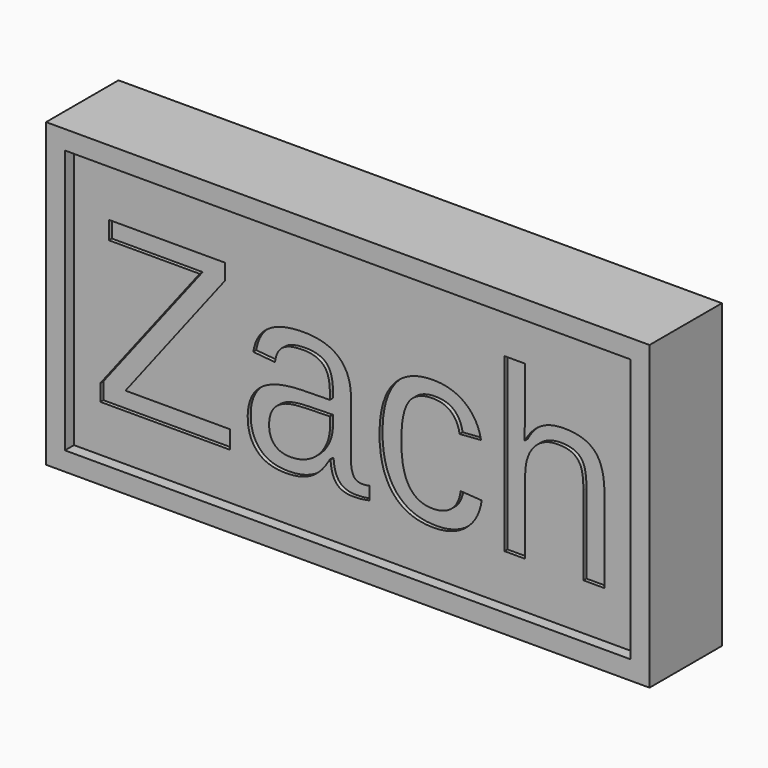
from build123d import *

# Parameters (mm, degrees)
F0_W          = 101.6
F0_H          = 50.8
F1_DEPTH      = 2.54
F1_DEPTH_BACK = 12.7
F2_TEXT_SIZE  = 39.9102132435
F3_DEPTH      = 25.4
F4_W          = 95.25
F4_H          = 44.45
F5_DEPTH      = 1.905


# Not quite as in the source:
# - Text() gives the source's letters only with a copy of the font that has no kerning and outlines rounded to 1/6400 em; it was checked with that copy


with BuildPart() as f1:
    # F0 (on Front) → F1 (new body, two sides)
    with BuildSketch(Plane.XZ) as f1_sk:
        Rectangle(F0_W, F0_H)
    extrude(amount=F1_DEPTH)
    extrude(f1_sk.sketch, amount=-F1_DEPTH_BACK)

    # F2 (on Front) → F3 (cut)
    with BuildSketch(Plane.XZ):
        with Locations((-44.45, -14.3716535354)):
            Text('Zach', F2_TEXT_SIZE, font='Arimo', text_align=(TextAlign.LEFT, TextAlign.BOTTOM))
    extrude(amount=F3_DEPTH, mode=Mode.SUBTRACT)

    # F4 (on face) → F5 (cut)
    with BuildSketch(Plane.XZ.offset(2.54)):
        Rectangle(F4_W, F4_H)
        Polygon((-21.3207842312, -14.3716535354), (-43.1840979237, -14.3716535354), (-43.1840979237, -11.5841745791), (-26.4654601571, 10.048408193), (-41.7622965769, 10.048408193), (-41.7622965769, 13.085325982), (-22.2312359708, 13.085325982), (-22.2312359708, 10.3789146465), (-38.9561097082, -11.3284997755), (-21.3207842312, -11.3284997755), align=None, mode=Mode.SUBTRACT)
        with BuildLine():
            add(Edge.make_bspline(
                [(2.1202300786, -14.2531700898), (2.0723865709, -14.2644539359), (2.0244889768, -14.2755061845), (1.9765384916, -14.2863264208), (1.928536319, -14.2969142632), (1.8804836712, -14.3072693632), (1.8323817688, -14.3173914054), (1.7842318409, -14.3272801075), (1.4515217244, -14.3939309898), (1.1653701807, -14.4427883458), (0.8778464225, -14.4834528728), (0.5892131652, -14.5159153346), (0.2997295795, -14.540208434), (0.0096509605, -14.5564035716), (-0.2807716037, -14.5646076058), (-0.5804951874, -14.5649707629), (-0.5896990689, -14.5649749573), (-0.5989026028, -14.564968796), (-0.6081053554, -14.5649498814), (-0.6173070643, -14.5649168171), (-0.6265076381, -14.5648692078), (-0.6357071562, -14.5648076595), (-0.7875369227, -14.5635882229), (-0.9299206082, -14.5592249002), (-1.0719768565, -14.5514039842), (-1.2135816903, -14.5398564949), (-1.3545676489, -14.5242863761), (-1.4947242147, -14.5043725712), (-1.6337982384, -14.4797711001), (-1.8578272202, -14.4315246626), (-1.9436101453, -14.4109477469), (-2.0287665222, -14.3882987845), (-2.1132065448, -14.3634883962), (-2.1968282954, -14.3364281893), (-2.2795188204, -14.3070335201), (-2.3611552078, -14.275226257), (-2.5664353754, -14.1877339842), (-2.688460794, -14.1285348762), (-2.8071174411, -14.0631063299), (-2.9218228133, -13.9912810865), (-3.031997384, -13.9129872601), (-3.1370889171, -13.8282820598), (-3.2366000922, -13.7373904914), (-3.3409652869, -13.6295411097), (-3.3517308662, -13.6182555071), (-3.3624156071, -13.6068928226), (-3.373018962, -13.5954536693), (-3.3835404086, -13.5839386813), (-3.3939794496, -13.5723485137), (-3.4043356129, -13.5606838426), (-3.4218631104, -13.5406556753), (-3.4290799143, -13.5323216241), (-3.4362718662, -13.5239468813), (-3.4434335167, -13.5155280025), (-3.4505647524, -13.5070634055), (-3.4576695392, -13.4985556697), (-3.4647441898, -13.4900034037), (-3.4950409567, -13.4530404598), (-3.5178814995, -13.4243094883), (-3.5403111831, -13.3952274423), (-3.5623310871, -13.3658060317), (-3.5839428285, -13.3360568326), (-3.6051485614, -13.305991288), (-3.6259509774, -13.2756207069), (-3.6918622823, -13.1765568465), (-3.7353793531, -13.1066963136), (-3.776940865, -13.0354960761), (-3.8165921512, -12.9630719356), (-3.8543855151, -12.8895328196), (-3.8903782144, -12.8149795142), (-3.9246304452, -12.7395033978), (-4.0727411922, -12.3924800864), (-4.1669573765, -12.1116367929), (-4.2430055331, -11.8236525092), (-4.3034622214, -11.5308576884), (-4.3504946413, -11.2349691554), (-4.3859181852, -10.9371065901), (-4.411209316, -10.6377955739), (-4.4275392817, -10.3369804153)],
                knots=[0, 0, 0, 0, 0, 0, 0, 0, 0, 0.042222485, 0.042222485, 0.042222485, 0.042222485, 0.042222485, 0.042222485, 0.042222485, 0.2914689848, 0.2914689848, 0.2914689848, 0.2914689848, 0.2914689848, 0.2914689848, 0.2914689848, 0.2993650731, 0.2993650731, 0.2993650731, 0.2993650731, 0.2993650731, 0.2993650731, 0.2993650731, 0.4217982218, 0.4217982218, 0.4217982218, 0.4217982218, 0.4217982218, 0.4217982218, 0.4217982218, 0.4985614805, 0.4985614805, 0.4985614805, 0.4985614805, 0.4985614805, 0.4985614805, 0.4985614805, 0.6176700118, 0.6176700118, 0.6176700118, 0.6176700118, 0.6176700118, 0.6176700118, 0.6176700118, 0.6314835454, 0.6314835454, 0.6314835454, 0.6314835454, 0.6314835454, 0.6314835454, 0.6314835454, 0.6412386363, 0.6412386363, 0.6412386363, 0.6412386363, 0.6412386363, 0.6412386363, 0.6412386363, 0.6734360167, 0.6734360167, 0.6734360167, 0.6734360167, 0.6734360167, 0.6734360167, 0.6734360167, 0.7452547743, 0.7452547743, 0.7452547743, 0.7452547743, 0.7452547743, 0.7452547743, 0.7452547743, 1, 1, 1, 1, 1, 1, 1, 1, 1], degree=8))
            Line((-4.4275392817, -10.3369804153), (-4.5397867565, -10.3369804153))
            add(Edge.make_bspline(
                [(-4.5397867565, -10.3369804153), (-4.6989322912, -10.6228529499), (-4.8654397559, -10.9044034311), (-5.0398569695, -11.1811167712), (-5.2227405504, -11.4522930031), (-5.4146542605, -11.7170482298), (-5.6161604317, -11.9743210252), (-5.8278044749, -12.222884286), (-6.2248736123, -12.6488737869), (-6.4062117551, -12.8301253263), (-6.5943114145, -13.0044098279), (-6.7893120016, -13.1709319529), (-6.9912707964, -13.328830089), (-7.2001355751, -13.4772116539), (-7.415706894, -13.6152019636), (-7.6570359382, -13.7531198692), (-7.6765314755, -13.764144601), (-7.6960724779, -13.7750884834), (-7.7156559173, -13.7859568656), (-7.7352799004, -13.7967528227), (-7.7549436687, -13.8074771555), (-7.7746475987, -13.8181283907), (-7.9598774687, -13.9173247981), (-8.128201701, -14.0007096611), (-8.299122184, -14.0788453561), (-8.4723974505, -14.1517600155), (-8.6477909922, -14.219515544), (-8.8250739729, -14.2822012454), (-9.0040279408, -14.3399274492), (-9.5238762569, -14.4923258297), (-9.8684372766, -14.5747052394), (-10.2168755023, -14.6408403527), (-10.5680927861, -14.6917652016), (-10.9211646192, -14.7285650748), (-11.27535199, -14.7523040322), (-11.6301084124, -14.7639797239), (-12.0218756536, -14.7645600126), (-12.0586689774, -14.7644909436), (-12.0954603852, -14.7642942673), (-12.1322485105, -14.7639667556), (-12.1690323301, -14.7635059918), (-12.2058111647, -14.7629103705), (-12.2425846784, -14.7621790975), (-12.5345795714, -14.7552945473), (-12.7894969276, -14.7426894188), (-13.0439357145, -14.7229772176), (-13.2976222781, -14.6955804767), (-13.5501788878, -14.6598670084), (-13.8011253191, -14.6151599852), (-14.0498816769, -14.5607549401), (-14.6146306709, -14.4118998696), (-14.9289650969, -14.3102803028), (-15.2368408008, -14.1896021011), (-15.5359927836, -14.0485311787), (-15.8239260589, -13.8860551788), (-16.0980677721, -13.7017524265), (-16.3559713585, -13.4961569042), (-16.6128105751, -13.2550363833), (-16.6299537809, -13.2387533032), (-16.6470023615, -13.2223700097), (-16.6639563168, -13.2058865029), (-16.6808156469, -13.1893027826), (-16.6975803516, -13.172618849), (-16.7142504311, -13.1558347021), (-16.7568553454, -13.1124357874), (-16.7826469414, -13.0856911595), (-16.8081535577, -13.0586644423), (-16.8334980747, -13.0314926807), (-16.8586387686, -13.0041371579), (-16.8835094255, -12.976531049), (-16.9081858959, -12.9487580261), (-16.9570325346, -12.892851997), (-16.9811987509, -12.864739711), (-17.0051294608, -12.8364434357), (-17.0288246643, -12.8079631711), (-17.0522843615, -12.7792989171), (-17.0755085523, -12.7504506737), (-17.0984972367, -12.721418441), (-17.3159498025, -12.4421984382), (-17.4934488294, -12.1786665008), (-17.6525223486, -11.9031487607), (-17.7927857656, -11.6173565933), (-17.9144687406, -11.3230633684), (-18.0182250134, -11.0220136334), (-18.1049783535, -10.7158485057), (-18.2288547833, -10.174000613), (-18.2729934659, -9.9398087085), (-18.3086871893, -9.7039682147), (-18.3364263663, -9.4669141452), (-18.3567025807, -9.2290167547), (-18.3699915597, -8.9905792432), (-18.3767418506, -8.7518362849), (-18.3775021855, -8.462315795), (-18.3773699876, -8.4116688612), (-18.3768975731, -8.3610500961), (-18.3761728169, -8.3104133112), (-18.3751037033, -8.2598075871), (-18.373746111, -8.2092028949), (-18.3720675156, -8.1586170557), (-18.3642410987, -7.9603123332), (-18.3556937454, -7.8127269586), (-18.3443214769, -7.6653539985), (-18.3300127044, -7.518265814), (-18.3126542658, -7.37154527), (-18.2921332324, -7.2252854886), (-18.2683387151, -7.0795896028), (-18.2204987187, -6.8242923929), (-18.1978791061, -6.7144064844), (-18.1732582368, -6.6049634059), (-18.14659107, -6.4960176867), (-18.117835032, -6.3876275118), (-18.0869509286, -6.2798544714), (-18.0539038566, -6.1727633102), (-17.9528626538, -5.8678550907), (-17.8794054874, -5.6718698998), (-17.7981089416, -5.4789460811), (-17.7088512486, -5.2895658518), (-17.6115891046, -5.1042052146), (-17.5063742257, -4.9233255043), (-17.3933699042, -4.7473649343), (-17.1649181121, -4.4238706014), (-17.0509306876, -4.2752555237), (-16.931108271, -4.1311761126), (-16.8057014629, -3.9918550847), (-16.6750010674, -3.8574535176), (-16.5393306752, -3.7280776971), (-16.399039247, -3.6037859647), (-16.2321705387, -3.4661881768), (-16.2097138083, -3.4478733565), (-16.1871055761, -3.4296558855), (-16.1643336387, -3.4115392681), (-16.1413915183, -3.3935257316), (-16.1182784625, -3.3756162258), (-16.0949994442, -3.3578104234), (-15.8756478875, -3.1920987159), (-15.6720707321, -3.0540746799), (-15.4618923027, -2.9257599984), (-15.2461040162, -2.8067398274), (-15.0255932629, -2.6965221894), (-14.8011169185, -2.594583727), (-14.5732852051, -2.500398113), (-13.7414786079, -2.1869294262), (-13.122166127, -2.0100504247), (-12.4912822413, -1.8726829294), (-11.8535568391, -1.7682016465), (-11.2123006813, -1.6911774216), (-10.56935838, -1.637504925), (-9.9252448993, -1.6038981033), (-9.2791245791, -1.5879133558)],
                knots=[0, 0, 0, 0, 0, 0, 0, 0, 0, 0.0806983163, 0.0806983163, 0.0806983163, 0.0806983163, 0.0806983163, 0.0806983163, 0.0806983163, 0.1441499828, 0.1441499828, 0.1441499828, 0.1441499828, 0.1441499828, 0.1441499828, 0.1441499828, 0.1497109072, 0.1497109072, 0.1497109072, 0.1497109072, 0.1497109072, 0.1497109072, 0.1497109072, 0.1963159919, 0.1963159919, 0.1963159919, 0.1963159919, 0.1963159919, 0.1963159919, 0.1963159919, 0.2839955127, 0.2839955127, 0.2839955127, 0.2839955127, 0.2839955127, 0.2839955127, 0.2839955127, 0.2930836196, 0.2930836196, 0.2930836196, 0.2930836196, 0.2930836196, 0.2930836196, 0.2930836196, 0.3561687707, 0.3561687707, 0.3561687707, 0.3561687707, 0.3561687707, 0.3561687707, 0.3561687707, 0.437974272, 0.437974272, 0.437974272, 0.437974272, 0.437974272, 0.437974272, 0.437974272, 0.4438596696, 0.4438596696, 0.4438596696, 0.4438596696, 0.4438596696, 0.4438596696, 0.4438596696, 0.4531018731, 0.4531018731, 0.4531018731, 0.4531018731, 0.4531018731, 0.4531018731, 0.4531018731, 0.4623277459, 0.4623277459, 0.4623277459, 0.4623277459, 0.4623277459, 0.4623277459, 0.4623277459, 0.5412737187, 0.5412737187, 0.5412737187, 0.5412737187, 0.5412737187, 0.5412737187, 0.5412737187, 0.6004056649, 0.6004056649, 0.6004056649, 0.6004056649, 0.6004056649, 0.6004056649, 0.6004056649, 0.612940254, 0.612940254, 0.612940254, 0.612940254, 0.612940254, 0.612940254, 0.612940254, 0.6495601002, 0.6495601002, 0.6495601002, 0.6495601002, 0.6495601002, 0.6495601002, 0.6495601002, 0.6774072449, 0.6774072449, 0.6774072449, 0.6774072449, 0.6774072449, 0.6774072449, 0.6774072449, 0.7294048701, 0.7294048701, 0.7294048701, 0.7294048701, 0.7294048701, 0.7294048701, 0.7294048701, 0.7759858343, 0.7759858343, 0.7759858343, 0.7759858343, 0.7759858343, 0.7759858343, 0.7759858343, 0.7831796509, 0.7831796509, 0.7831796509, 0.7831796509, 0.7831796509, 0.7831796509, 0.7831796509, 0.8433220064, 0.8433220064, 0.8433220064, 0.8433220064, 0.8433220064, 0.8433220064, 0.8433220064, 1, 1, 1, 1, 1, 1, 1, 1, 1], degree=8))
            Line((-9.2791245791, -1.5879133558), (-4.5397867565, -1.5068457351))
            Line((-4.5397867565, -1.5068457351), (-4.5397867565, -0.3594271044))
            add(Edge.make_bspline(
                [(-4.5397867565, -0.3594271044), (-4.5397867565, -0.0471676373), (-4.5489979223, 0.2642359035), (-4.5686031467, 0.5749227047), (-4.6001212331, 0.8844814896), (-4.6454491159, 1.1919380206), (-4.7068755731, 1.4957530331), (-4.7871520165, 1.7938076316), (-4.9181552502, 2.1636755062), (-4.9483063929, 2.2433071624), (-4.9802244631, 2.322176084), (-5.0139746362, 2.4001998871), (-5.0496203492, 2.4772868135), (-5.0872214791, 2.5533366776), (-5.1268325216, 2.6282418129), (-5.2156943707, 2.7852999699), (-5.2655285444, 2.8670995474), (-5.3180669747, 2.9471143586), (-5.3733603548, 3.0251613571), (-5.4314402552, 3.1010517784), (-5.4923129925, 3.1745960743), (-5.5559534985, 3.2456088475), (-5.6310296562, 3.3229020724), (-5.6398067111, 3.3318440793), (-5.6486287799, 3.340741653), (-5.6574947027, 3.3495960083), (-5.6664037329, 3.3584077294), (-5.675355538, 3.3671767697), (-5.6843501985, 3.3759024515), (-5.7636980826, 3.4521161479), (-5.8366010364, 3.5169933585), (-5.9119590925, 3.579130179), (-5.9896221416, 3.6384751387), (-6.0694313269, 3.6950058711), (-6.1512224279, 3.7487247692), (-6.234829244, 3.7996546403), (-6.411711238, 3.8996118496), (-6.5052464455, 3.948215665), (-6.6004984184, 3.9936998142), (-6.6972814534, 4.0361416364), (-6.7954217859, 4.075634546), (-6.8947603861, 4.1122821546), (-6.9951550912, 4.1461937719), (-7.2072694675, 4.2116899615), (-7.3191661137, 4.2427598664), (-7.4320142638, 4.2708395201), (-7.5456726196, 4.2960760162), (-7.660016813, 4.318613329), (-7.774939886, 4.3385906211), (-7.89035277, 4.3561405506), (-8.069475185, 4.3797185313), (-8.132889357, 4.3873618195), (-8.1964149556, 4.3943377406), (-8.260040567, 4.400665895), (-8.3237556896, 4.4063651853), (-8.387550734, 4.4114538174), (-8.4514170232, 4.4159492999), (-8.5488134223, 4.4219200792), (-8.5822974051, 4.4238137742), (-8.6157976036, 4.4255519411), (-8.6493129302, 4.4271369424), (-8.6828423459, 4.4285710909), (-8.716384861, 4.42985665), (-8.7499395347, 4.4309958336), (-8.8016844468, 4.4325296732), (-8.8199093956, 4.4330275055), (-8.8381803217, 4.433484303), (-8.8564972252, 4.4339000658), (-8.8748601059, 4.4342747939), (-8.8932689639, 4.4346084872), (-8.9117237992, 4.4349011458), (-8.9488732168, 4.4354064036), (-8.9675238162, 4.4356200013), (-8.9861773027, 4.4357905718), (-9.0048339878, 4.4359169613), (-9.0234936022, 4.4359998533), (-9.0421552956, 4.4360417685), (-9.0608176369, 4.436047065), (-9.3963556285, 4.4355952628), (-9.7121008241, 4.4268411998), (-10.0270096867, 4.4086407965), (-10.3407737687, 4.3794945282), (-10.6524864039, 4.3375228228), (-10.9605843501, 4.2802659949), (-11.2628606398, 4.2047091523), (-11.6807139591, 4.0646341008), (-11.8034771274, 4.0188409764), (-11.9242497025, 3.9686665118), (-12.0426562647, 3.9137855811), (-12.1582253189, 3.8538708827), (-12.2704007797, 3.7886121321), (-12.3785614227, 3.717747881), (-12.4949216056, 3.6315765485), (-12.5077040891, 3.6219606466), (-12.5204334418, 3.6122802321), (-12.5330761333, 3.6025122172), (-12.5456615048, 3.592671522), (-12.5581736935, 3.5827496445), (-12.5706174936, 3.5727506046), (-12.5963832696, 3.5517681823), (-12.6096999236, 3.5407661866), (-12.6229381032, 3.5296703841), (-12.6360970603, 3.518481263), (-12.6491760685, 3.5071993392), (-12.6621744232, 3.4958251564), (-12.6750914415, 3.4843592859), (-12.8240209367, 3.350259612), (-12.9509426698, 3.2174342306), (-13.067765377, 3.0751416504), (-13.1741013058, 2.9244168942), (-13.2699551708, 2.7664099424), (-13.3556030924, 2.6022983985), (-13.4314965398, 2.4332174175), (-13.5524456061, 2.1194676101), (-13.6006409227, 1.9760548888), (-13.6431050139, 1.8304227439), (-13.6801866898, 1.6829753731), (-13.7122370593, 1.5340610979), (-13.7395959063, 1.3839679992), (-13.7625831677, 1.2329212513), (-13.7814955107, 1.0810821549)],
                knots=[0, 0, 0, 0, 0, 0, 0, 0, 0, 0.1739467518, 0.1739467518, 0.1739467518, 0.1739467518, 0.1739467518, 0.1739467518, 0.1739467518, 0.2222010183, 0.2222010183, 0.2222010183, 0.2222010183, 0.2222010183, 0.2222010183, 0.2222010183, 0.276853969, 0.276853969, 0.276853969, 0.276853969, 0.276853969, 0.276853969, 0.276853969, 0.284045782, 0.284045782, 0.284045782, 0.284045782, 0.284045782, 0.284045782, 0.284045782, 0.3399934326, 0.3399934326, 0.3399934326, 0.3399934326, 0.3399934326, 0.3399934326, 0.3399934326, 0.4001189113, 0.4001189113, 0.4001189113, 0.4001189113, 0.4001189113, 0.4001189113, 0.4001189113, 0.4658580156, 0.4658580156, 0.4658580156, 0.4658580156, 0.4658580156, 0.4658580156, 0.4658580156, 0.5017777582, 0.5017777582, 0.5017777582, 0.5017777582, 0.5017777582, 0.5017777582, 0.5017777582, 0.5205814042, 0.5205814042, 0.5205814042, 0.5205814042, 0.5205814042, 0.5205814042, 0.5205814042, 0.5307652673, 0.5307652673, 0.5307652673, 0.5307652673, 0.5307652673, 0.5307652673, 0.5307652673, 0.5410304835, 0.5410304835, 0.5410304835, 0.5410304835, 0.5410304835, 0.5410304835, 0.5410304835, 0.7153413481, 0.7153413481, 0.7153413481, 0.7153413481, 0.7153413481, 0.7153413481, 0.7153413481, 0.7893007125, 0.7893007125, 0.7893007125, 0.7893007125, 0.7893007125, 0.7893007125, 0.7893007125, 0.7985009261, 0.7985009261, 0.7985009261, 0.7985009261, 0.7985009261, 0.7985009261, 0.7985009261, 0.8084618671, 0.8084618671, 0.8084618671, 0.8084618671, 0.8084618671, 0.8084618671, 0.8084618671, 0.9140814124, 0.9140814124, 0.9140814124, 0.9140814124, 0.9140814124, 0.9140814124, 0.9140814124, 1, 1, 1, 1, 1, 1, 1, 1, 1], degree=8))
            Line((-13.7814955107, 1.0810821549), (-17.4420103816, 1.4115886083))
            add(Edge.make_bspline(
                [(-17.4420103816, 1.4115886083), (-17.4108096201, 1.6094101029), (-17.3744287629, 1.8063258743), (-17.3326011139, 2.0021298742), (-17.285053635, 2.1965711866), (-17.2315203531, 2.389357789), (-17.1717557665, 2.5801603145), (-17.0713765056, 2.8658835243), (-17.0354888839, 2.9625249929), (-16.997856966, 3.0584893833), (-16.9584550801, 3.1537234177), (-16.9172611247, 3.2481717315), (-16.8742573899, 3.3417772274), (-16.7380588984, 3.6234478963), (-16.6391045569, 3.8086908156), (-16.532474393, 3.9896835867), (-16.4181547836, 4.165915709), (-16.296231026, 4.3369049972), (-16.1669059216, 4.5022097971), (-15.8311666563, 4.8941827389), (-15.6166482636, 5.1140404217), (-15.388050535, 5.3197207821), (-15.1467700802, 5.5105873799), (-14.8943822827, 5.6864987961), (-14.6325289754, 5.8476708305), (-14.1966232294, 6.0850826999), (-14.0273996943, 6.1702017989), (-13.8554895956, 6.2500458129), (-13.681206612, 6.3247732099), (-13.504837434, 6.3945651577), (-13.3266370254, 6.4596153704), (-12.5818340863, 6.7102310481), (-12.0016258405, 6.8552304044), (-11.411874895, 6.9618334449), (-10.8168361705, 7.0357796445), (-10.2193479515, 7.0818594903), (-9.6208360761, 7.10394144), (-8.9904386222, 7.1050533468), (-8.9595579831, 7.1050526019), (-8.9286777869, 7.1049902982), (-8.8977990821, 7.1048623254), (-8.8669223882, 7.1046668113), (-8.8360476954, 7.1044041213), (-8.3448625684, 7.0991974595), (-7.8851490858, 7.0795860157), (-7.4263295563, 7.0434952693), (-6.9692935129, 6.9888012836), (-6.5155266288, 6.9129962275), (-6.0671056661, 6.8132171862), (-5.2181558439, 6.5685935892), (-4.8164334569, 6.4275134985), (-4.4241708931, 6.2606919963), (-4.0448967164, 6.065864476), (-3.6827846779, 5.8412847055), (-3.3422562439, 5.5864138371), (-3.0048084716, 5.2831103032), (-2.9825183716, 5.2628120698), (-2.9603521248, 5.2423795759), (-2.9383098198, 5.2218149353), (-2.9163950712, 5.2011159294), (-2.8946110064, 5.1802808128), (-2.8041463681, 5.0926864286), (-2.7366505735, 5.0247127045), (-2.6705114427, 4.9554110294), (-2.6057681559, 4.8848045019), (-2.5424565, 4.8129202371), (-2.4806088685, 4.7397893663), (-2.1707745443, 4.3581481574), (-1.9466979943, 4.0300217078), (-1.7503923764, 3.6838889991), (-1.5822039361, 3.3230113187), (-1.441204543, 2.9507236729), (-1.3257519025, 2.5701557672), (-1.1614513855, 1.8797691406), (-1.1036296929, 1.5718716954), (-1.0593902946, 1.2613980901), (-1.0276718987, 0.9492260493), (-1.0074435626, 0.6360489504), (-0.9977553311, 0.3223689597), (-0.9977553311, 0.008495174)],
                knots=[0, 0, 0, 0, 0, 0, 0, 0, 0.0596367309, 0.0596367309, 0.0596367309, 0.0596367309, 0.0596367309, 0.0596367309, 0.0904170918, 0.0904170918, 0.0904170918, 0.0904170918, 0.0904170918, 0.0904170918, 0.1531591885, 0.1531591885, 0.1531591885, 0.1531591885, 0.1531591885, 0.1531591885, 0.2448665518, 0.2448665518, 0.2448665518, 0.2448665518, 0.2448665518, 0.2448665518, 0.3013796914, 0.3013796914, 0.3013796914, 0.3013796914, 0.3013796914, 0.3013796914, 0.4789492906, 0.4789492906, 0.4789492906, 0.4789492906, 0.4789492906, 0.4789492906, 0.4880954074, 0.4880954074, 0.4880954074, 0.4880954074, 0.4880954074, 0.4880954074, 0.624461649, 0.624461649, 0.624461649, 0.624461649, 0.624461649, 0.624461649, 0.7509541431, 0.7509541431, 0.7509541431, 0.7509541431, 0.7509541431, 0.7509541431, 0.759957006, 0.759957006, 0.759957006, 0.759957006, 0.759957006, 0.759957006, 0.788564395, 0.788564395, 0.788564395, 0.788564395, 0.788564395, 0.788564395, 0.9068149086, 0.9068149086, 0.9068149086, 0.9068149086, 0.9068149086, 0.9068149086, 1, 1, 1, 1, 1, 1, 1, 1], degree=7))
            Line((-0.9977553311, 0.008495174), (-0.9977553311, -9.0710783389))
            add(Edge.make_bspline(
                [(-0.9977553311, -9.0710783389), (-0.9977553311, -9.4015975179), (-0.9869638809, -9.7248294826), (-0.9638658313, -10.0396751559), (-0.9265089998, -10.3438928282), (-0.872574118, -10.6341638877), (-0.7993915889, -10.9061046653), (-0.6966775194, -11.1747143201), (-0.6888558637, -11.1946428274), (-0.6808910824, -11.2144134641), (-0.6727819908, -11.2340232835), (-0.6645274372, -11.253469305), (-0.6561263029, -11.2727485139), (-0.6433613064, -11.30128243), (-0.639109193, -11.3106656824), (-0.6348210326, -11.3200072531), (-0.6304966981, -11.3293067756), (-0.6261360649, -11.3385638818), (-0.6217390113, -11.3477782019), (-0.6150983117, -11.3615149013), (-0.6128837365, -11.3660664611), (-0.6106616923, -11.3706040448), (-0.6084321791, -11.3751276522), (-0.6061951968, -11.3796372835), (-0.6039507454, -11.3841329385), (-0.5994469044, -11.3930962965), (-0.5971871974, -11.397563934), (-0.5949202416, -11.4020176398), (-0.5926462253, -11.4064574528), (-0.5903649872, -11.4108833413), (-0.5880760168, -11.4152952031), (-0.5540656724, -11.4803928836), (-0.5195891888, -11.5387862009), (-0.4823236411, -11.5947318328), (-0.4422642465, -11.6481023093), (-0.39942984, -11.6987865408), (-0.3538659114, -11.7466926844), (-0.2259491542, -11.8662265277), (-0.1389769165, -11.9329426263), (-0.0450828962, -11.9915572995), (0.0552382648, -12.0419900556), (0.1613953048, -12.0843610209), (0.2727417144, -12.1189366084), (0.4543187889, -12.1614748474), (0.5214911704, -12.1744811376), (0.5900184977, -12.1851682343), (0.659793238, -12.193612434), (0.7307130936, -12.1998956645), (0.8026826968, -12.204102431), (0.8849507449, -12.2066001979), (0.8943162313, -12.2068514239), (0.9037117637, -12.2070704396), (0.9131373421, -12.207257245), (0.9225929665, -12.2074118401), (0.9320786368, -12.207534225), (0.9503546419, -12.2077074153), (0.9591279199, -12.207762156), (0.9679130046, -12.2077947348), (0.9767128753, -12.2077872161), (0.9855226119, -12.2077679489), (0.9943449409, -12.2077199491), (1.1548821853, -12.2064250884), (1.3100245207, -12.1981283209), (1.4680357048, -12.1833757861), (1.6284241242, -12.1627479), (1.7907830937, -12.1367725632), (1.9547945513, -12.1059160467), (2.1202300786, -12.070580303)],
                knots=[0, 0, 0, 0, 0, 0, 0, 0, 0.3668322722, 0.3668322722, 0.3668322722, 0.3668322722, 0.3668322722, 0.3668322722, 0.3964760825, 0.3964760825, 0.3964760825, 0.3964760825, 0.3964760825, 0.3964760825, 0.411096159, 0.411096159, 0.411096159, 0.411096159, 0.411096159, 0.411096159, 0.4183742417, 0.4183742417, 0.4183742417, 0.4183742417, 0.4183742417, 0.4183742417, 0.4256523248, 0.4256523248, 0.4256523248, 0.4256523248, 0.4256523248, 0.4256523248, 0.5261102012, 0.5261102012, 0.5261102012, 0.5261102012, 0.5261102012, 0.5261102012, 0.6921539296, 0.6921539296, 0.6921539296, 0.6921539296, 0.6921539296, 0.6921539296, 0.7863117125, 0.7863117125, 0.7863117125, 0.7863117125, 0.7863117125, 0.7863117125, 0.7983639948, 0.7983639948, 0.7983639948, 0.7983639948, 0.7983639948, 0.7983639948, 0.8094594784, 0.8094594784, 0.8094594784, 0.8094594784, 0.8094594784, 0.8094594784, 1, 1, 1, 1, 1, 1, 1, 1], degree=7))
            Line((2.1202300786, -12.070580303), (2.1202300786, -14.2531700898))
        make_face(mode=Mode.SUBTRACT)
        with BuildLine():
            add(Edge.make_bspline(
                [(21.0214576319, -8.0982668911), (20.9957071096, -8.2911977273), (20.96547661, -8.4834668163), (20.9305977042, -8.6749247547), (20.8909047221, -8.8654014273), (20.8462414218, -9.0547075619), (20.7964676582, -9.2426362839), (20.6484089602, -9.744213245), (20.5403650651, -10.0549565107), (20.4167893684, -10.3599982233), (20.2773340718, -10.658117743), (20.1219260213, -10.9481077219), (19.9508521903, -11.2288150806), (19.6085193908, -11.72643384), (19.4416024852, -11.9464363526), (19.2645231023, -12.1585737913), (19.0778305554, -12.362408378), (18.8821758178, -12.5576591735), (18.6782844856, -12.7441776758), (18.4157398294, -12.9649732606), (18.3641122237, -13.007510966), (18.3120431248, -13.0495030215), (18.259536495, -13.0909398125), (18.2066000728, -13.1318225367), (18.1532413893, -13.1721501202), (18.0458182848, -13.2515644855), (17.9917910274, -13.2906319259), (17.9373820124, -13.3291084544), (17.8825912399, -13.366994071), (17.8274187099, -13.4042887756), (17.7718644224, -13.4409925684), (17.3122632223, -13.7377157874), (16.8885801236, -13.9676410858), (16.4479971623, -14.1648112317), (15.9938610788, -14.3290608316), (15.5295025803, -14.4614823151), (15.0580403377, -14.5639175888), (14.4598493241, -14.6577946118), (14.3371546357, -14.6751677071), (14.2141890311, -14.6907452948), (14.0909894007, -14.7045663214), (13.9675900457, -14.7166704981), (13.8440226247, -14.7270978858), (13.6613703154, -14.7400771726), (13.6021935916, -14.7439083991), (13.5427859281, -14.7473821605), (13.4831473249, -14.7504984566), (13.4232777819, -14.7532572874), (13.3631772991, -14.7556586531), (13.2330909043, -14.7600657037), (13.163314022, -14.7619506755), (13.0935154411, -14.7633472702), (13.0236984126, -14.7642576768), (12.9538692266, -14.7646964712), (12.8840372131, -14.7646906169), (12.4684098944, -14.7622431792), (12.1228565109, -14.7500956931), (11.7778871456, -14.727071879), (11.433981896, -14.6923435092), (11.0917661156, -14.6450385428), (10.7520048095, -14.5842839661), (10.2536469503, -14.4731618595), (10.0924828331, -14.4337489272), (9.9322060574, -14.390945097), (9.772930516, -14.3446665108), (9.6147784005, -14.2948366339), (9.4578793019, -14.2413891432), (9.0132319275, -14.0780715685), (8.7288478145, -13.9591643931), (8.4501640936, -13.8272274682), (8.1781272611, -13.6820888414), (7.9136557824, -13.5237765444), (7.6576126847, -13.3525687081), (7.2109312786, -13.0204546501), (7.0170870091, -12.8637666102), (6.8296537985, -12.6992749559), (6.6489347385, -12.5273497736), (6.475139172, -12.3484235385), (6.308394309, -12.1629788167), (6.1116139589, -11.9269929159), (6.0748154835, -11.8820697454), (6.0383619056, -11.8367664133), (6.0022535154, -11.7910828956), (5.966490404, -11.7450191858), (5.9310724641, -11.6985752942), (5.6174576843, -11.2798862315), (5.3642737261, -10.8888416991), (5.1367964735, -10.4815538395), (4.934278985, -10.0609825582), (4.7554001971, -9.6298363036), (4.5986044906, -9.1903942147), (4.255719932, -8.0688623856), (4.0962273564, -7.3787075342), (3.9777086178, -6.6791111913), (3.8947314509, -5.9740333651), (3.8426468734, -5.2662180433), (3.8175798606, -4.5571949518), (3.8162939352, -3.7523818306), (3.816569721, -3.6574847899), (3.8172864111, -3.5626002899), (3.818452133, -3.4677317391), (3.8200727821, -3.3728771507), (3.8221551591, -3.2780363692), (3.8408864373, -2.5828899043), (3.8759688467, -1.9835956927), (3.9320833566, -1.3858094859), (4.0117637177, -0.7906815914), (4.1179542465, -0.2000406153), (4.2539566214, 0.3836162768), (4.5756886032, 1.4731181921), (4.7550567179, 1.9808903384), (4.9638788628, 2.4777393941), (5.2044898581, 2.9600992544), (5.4787421684, 3.4237599034), (5.7874153784, 3.8641934898), (6.1708693597, 4.3276585253), (6.2131400262, 4.3777439287), (6.2558883224, 4.4274169359), (6.2991123956, 4.4766691699), (6.3428158396, 4.5254894429), (6.3870004383, 4.5738674536), (6.5729411713, 4.7734297019), (6.7189880104, 4.9205739048), (6.8697304434, 5.0629478077), (7.0250649128, 5.2002930898), (7.184849562, 5.3323796153), (7.3489005104, 5.4590096526), (7.7682565508, 5.7609194495), (8.0285898591, 5.9292952904), (8.2971956268, 6.0845814486), (8.5732030059, 6.2265119916), (8.8556894164, 6.3550726054), (9.1437072351, 6.4704499766), (9.5863471854, 6.6255555828), (9.737602475, 6.6747569561), (9.8899586267, 6.7206333029), (10.0433034477, 6.7632434416), (10.197530967, 6.8026546907), (10.3525421224, 6.8389405576), (10.8293536303, 6.9407251468), (11.1533853028, 6.9963040886), (11.4795705715, 7.0396057069), (11.8072479914, 7.0713787365), (12.13587151, 7.0923759706), (12.4650149409, 7.1033184713), (12.8638312364, 7.1052071445), (12.9332953841, 7.1051190007), (13.0027550689, 7.1045863575), (13.0722017147, 7.1035897924), (13.1416295122, 7.1021178879), (13.2110354193, 7.100167231), (13.4791054717, 7.0907987408), (13.6775945533, 7.0799137825), (13.8757876944, 7.0649237617), (14.0735684392, 7.0456607845), (14.2708030701, 7.0219567783), (14.4673410885, 6.9936474308), (15.1255516889, 6.882402124), (15.5835714977, 6.7775685592), (16.0344479384, 6.6440190281), (16.4752259164, 6.4800611096), (16.9027607638, 6.284705513), (17.3139014224, 6.0581291202), (17.7731714669, 5.7582132857), (17.8400528012, 5.7132958573), (17.9063624784, 5.6675096392), (17.9721004984, 5.6208546314), (18.0372668611, 5.5733308338), (18.1018615667, 5.5249382464), (18.2123025479, 5.4399614303), (18.2583903224, 5.4038131999), (18.3041421726, 5.3672414624), (18.3495519139, 5.3302523036), (18.3946129435, 5.2928486111), (18.4393182403, 5.2550300739), (18.6254326301, 5.0945407937), (18.7634992071, 4.9680361747), (18.8976303172, 4.8373304915), (19.0276142935, 4.7025027859), (19.1532604605, 4.5636627488), (19.2744020122, 4.4209534935), (19.7305989796, 3.8476604123), (20.0309632978, 3.3891951365), (20.288024964, 2.9040814705), (20.501737648, 2.3979777565), (20.6742857966, 1.8765052967), (20.8089046654, 1.3447016216), (20.9092101571, 0.8066994388)],
                knots=[0, 0, 0, 0, 0, 0, 0, 0, 0.0252018397, 0.0252018397, 0.0252018397, 0.0252018397, 0.0252018397, 0.0252018397, 0.0678407751, 0.0678407751, 0.0678407751, 0.0678407751, 0.0678407751, 0.0678407751, 0.1036791817, 0.1036791817, 0.1036791817, 0.1036791817, 0.1036791817, 0.1036791817, 0.1123592084, 0.1123592084, 0.1123592084, 0.1123592084, 0.1123592084, 0.1123592084, 0.1210179126, 0.1210179126, 0.1210179126, 0.1210179126, 0.1210179126, 0.1210179126, 0.1835038674, 0.1835038674, 0.1835038674, 0.1835038674, 0.1835038674, 0.1835038674, 0.1995761575, 0.1995761575, 0.1995761575, 0.1995761575, 0.1995761575, 0.1995761575, 0.2072345549, 0.2072345549, 0.2072345549, 0.2072345549, 0.2072345549, 0.2072345549, 0.2160891663, 0.2160891663, 0.2160891663, 0.2160891663, 0.2160891663, 0.2160891663, 0.2599427777, 0.2599427777, 0.2599427777, 0.2599427777, 0.2599427777, 0.2599427777, 0.2810537057, 0.2810537057, 0.2810537057, 0.2810537057, 0.2810537057, 0.2810537057, 0.3203049366, 0.3203049366, 0.3203049366, 0.3203049366, 0.3203049366, 0.3203049366, 0.3520842649, 0.3520842649, 0.3520842649, 0.3520842649, 0.3520842649, 0.3520842649, 0.3594783681, 0.3594783681, 0.3594783681, 0.3594783681, 0.3594783681, 0.3594783681, 0.4182005115, 0.4182005115, 0.4182005115, 0.4182005115, 0.4182005115, 0.4182005115, 0.5071541223, 0.5071541223, 0.5071541223, 0.5071541223, 0.5071541223, 0.5071541223, 0.5190443761, 0.5190443761, 0.5190443761, 0.5190443761, 0.5190443761, 0.5190443761, 0.5943259854, 0.5943259854, 0.5943259854, 0.5943259854, 0.5943259854, 0.5943259854, 0.6620529194, 0.6620529194, 0.6620529194, 0.6620529194, 0.6620529194, 0.6620529194, 0.6703342522, 0.6703342522, 0.6703342522, 0.6703342522, 0.6703342522, 0.6703342522, 0.6965332102, 0.6965332102, 0.6965332102, 0.6965332102, 0.6965332102, 0.6965332102, 0.7356971352, 0.7356971352, 0.7356971352, 0.7356971352, 0.7356971352, 0.7356971352, 0.7557790244, 0.7557790244, 0.7557790244, 0.7557790244, 0.7557790244, 0.7557790244, 0.7971940612, 0.7971940612, 0.7971940612, 0.7971940612, 0.7971940612, 0.7971940612, 0.8059279201, 0.8059279201, 0.8059279201, 0.8059279201, 0.8059279201, 0.8059279201, 0.8309380761, 0.8309380761, 0.8309380761, 0.8309380761, 0.8309380761, 0.8309380761, 0.8900571275, 0.8900571275, 0.8900571275, 0.8900571275, 0.8900571275, 0.8900571275, 0.9002347266, 0.9002347266, 0.9002347266, 0.9002347266, 0.9002347266, 0.9002347266, 0.9076136803, 0.9076136803, 0.9076136803, 0.9076136803, 0.9076136803, 0.9076136803, 0.9312059413, 0.9312059413, 0.9312059413, 0.9312059413, 0.9312059413, 0.9312059413, 1, 1, 1, 1, 1, 1, 1, 1], degree=7))
            Line((20.9092101571, 0.8066994388), (17.2985830527, 0.5385526936))
            add(Edge.make_bspline(
                [(17.2985830527, 0.5385526936), (17.2791265024, 0.6656989877), (17.2568850482, 0.7922640525), (17.2317478013, 0.918156184), (17.2036025451, 1.0432700011), (17.1723388134, 1.167487391), (17.1378509687, 1.2906784545), (17.1000412802, 1.4127024517), (16.9909073025, 1.732297517), (16.9137140626, 1.9276785643), (16.8268777022, 2.1187837546), (16.730128266, 2.3048230848), (16.6233300179, 2.4850080614), (16.506525188, 2.658577858), (16.3799828695, 2.8248282539), (16.2240020313, 3.0067641425), (16.2035453235, 3.0302096193), (16.1828829457, 3.0534797832), (16.1620148979, 3.0765746344), (16.14094118, 3.0994941728), (16.1196617922, 3.1222383983), (16.0981767344, 3.1448073111), (16.0523264184, 3.1921433728), (16.0279306555, 3.2168606121), (16.0032857794, 3.2413282485), (15.978402743, 3.2655612621), (15.9532973214, 3.2895765627), (15.9279733548, 3.3133685495), (15.902408303, 3.3368976614), (15.7066170202, 3.5124572339), (15.5246354564, 3.6514998405), (15.3318603331, 3.7760784065), (15.1297799564, 3.885864933), (14.9199712341, 3.9810998925), (14.7039885185, 4.0623932682), (14.4832770828, 4.1305714954), (14.0770247874, 4.2320572653), (13.8925514908, 4.2695349073), (13.7062230871, 4.2995254045), (13.5185001355, 4.3225598077), (13.3297676597, 4.3391551313), (13.1403320897, 4.349797929), (12.9504194939, 4.3549343561), (12.7095380575, 4.3549753314), (12.6589165498, 4.3546336644), (12.6083233256, 4.3539381277), (12.5577521242, 4.3528791415), (12.5072088173, 4.3514506029), (12.4567020264, 4.3496470414), (12.4062298332, 4.3474595915), (12.2108566588, 4.3374734097), (12.0662570465, 4.3268400286), (11.9220936759, 4.3128117746), (11.7784832354, 4.2952087114), (11.6355649139, 4.2738451145), (11.4934995237, 4.2485336248), (11.3524686238, 4.2190894023), (11.129069364, 4.1651470551), (11.0459089432, 4.143418508), (10.9632368475, 4.1201113055), (10.8811008642, 4.0951894294), (10.7995518111, 4.0686189686), (10.7186432467, 4.0403689113), (10.63843118, 4.0104119366), (10.4119561436, 3.9200962042), (10.2674959613, 3.8555348444), (10.1259945734, 3.7849066004), (9.98785185, 3.708127446), (9.8534574537, 3.6251779982), (9.7231821031, 3.5361176601), (9.597368835, 3.4410987628), (9.3697008529, 3.2516621226), (9.2667557181, 3.1585034203), (9.1676976184, 3.0610762788), (9.0726780398, 2.9595865442), (8.981797243, 2.8542686011), (8.8951103083, 2.7453797419), (8.8126331791, 2.6331945365), (8.7111659458, 2.4838858469), (8.6882195076, 2.4493207612), (8.6655409401, 2.4142240906), (8.64309445, 2.3786528492), (8.6208852928, 2.3425919014), (8.5989302869, 2.3060102641), (8.577212722, 2.2689468955), (8.4842265462, 2.1062800893), (8.4169717031, 1.9783873003), (8.3537420502, 1.8480764824), (8.2943058942, 1.7156707663), (8.2384389207, 1.5814507292), (8.1859259124, 1.445653422), (8.1365624673, 1.3084713965), (7.9401356608, 0.7225670169), (7.8212954489, 0.2629637084), (7.7266820816, -0.2044988583), (7.6521930311, -0.6769553967), (7.59447842, -1.1523800566), (7.5511028284, -1.6296448367), (7.5200854821, -2.1083774915), (7.4940048113, -2.7304171293), (7.4890185907, -2.8719458869), (7.4849372892, -3.013559368), (7.4817249566, -3.1552471153), (7.4793482179, -3.2969997612), (7.4777760048, -3.4388090056), (7.476979288, -3.5806675935), (7.4769060342, -3.7950843723), (7.4770953866, -3.8675962273), (7.4775208739, -3.9400911353), (7.4781807534, -4.0125721843), (7.4790726156, -4.0850429073), (7.4802028938, -4.1575005329), (7.4815827956, -4.2299388542), (7.4939071998, -4.7782380903), (7.5153724989, -5.2530066656), (7.5488791873, -5.7267116973), (7.5960180849, -6.1989447252), (7.6587270667, -6.6688393206), (7.7394244668, -7.1350406533), (7.8410740993, -7.5956943059), (8.0381372171, -8.299618307), (8.1161640002, -8.5482655482), (8.2025515812, -8.7938441284), (8.2980415681, -9.0357012258), (8.4034151248, -9.2729612565), (8.519474101, -9.5045355343), (8.646999825, -9.7291432265), (8.8094665757, -9.980647842), (8.8325890552, -10.0157133505), (8.8560221591, -10.050559156), (8.8797709852, -10.085175931), (8.9038419539, -10.1195530363), (8.9282354273, -10.1536852802), (8.9529480909, -10.1875707275), (9.0027289161, -10.2544345746), (9.027709671, -10.2873139068), (9.052927367, -10.3198375537), (9.078382004, -10.3520055156), (9.104073582, -10.3838177922), (9.1300021011, -10.4152743837), (9.1561675612, -10.4463752901), (9.2780424618, -10.5882968808), (9.377521805, -10.6958804043), (9.4809895788, -10.7995747652), (9.5883944723, -10.8991000746), (9.6996468778, -10.994199118), (9.8146134929, -11.0846436028), (9.9331119216, -11.1702404059), (10.1734220507, -11.3292669407), (10.2950784025, -11.4029749819), (10.4196588209, -11.4718201192), (10.5469328428, -11.5357197445), (10.6766583078, -11.5946439116), (10.8085846132, -11.6486087815), (10.9424559694, -11.6976700675), (11.1486326485, -11.7649662237), (11.2197122707, -11.786710529), (11.2912194325, -11.8071624852), (11.3631211027, -11.8263377187), (11.4353854141, -11.8442540321), (11.50798177, -11.8609310431), (11.5808809501, -11.8763898231), (11.793008563, -11.9177365335), (11.9329505248, -11.9405066226), (12.073696122, -11.959117151), (12.2150779769, -11.9737340895), (12.3569470362, -11.9845302656), (12.4991732922, -11.9916805963), (12.6416465033, -11.9953573214), (12.8167902822, -11.9958091053), (12.8493046469, -11.9957204034), (12.881814218, -11.9954562818), (12.9143146498, -11.9950142023), (12.946803043, -11.9943919371), (12.9792779439, -11.9935875693), (13.0117393451, -11.9925994929), (13.1421170241, -11.9878861929), (13.2399186898, -11.982657248), (13.3375576654, -11.975687856), (13.4349938118, -11.9669260535), (13.5321829824, -11.9563204281), (13.6290771368, -11.9438209119), (13.7256244559, -11.9293795737), (14.0373412049, -11.8761169701), (14.2509692185, -11.8292808741), (14.461933238, -11.7719404135), (14.6694711573, -11.7036849176), (14.8727963101, -11.6242393268), (15.0711168714, -11.5335139213), (15.2636573735, -11.4316602077), (15.4874178425, -11.2963066039), (15.5248866175, -11.2730402031), (15.56208866, -11.2493337613), (15.5990239699, -11.2251872784), (15.6356925472, -11.2006007545), (15.6720943919, -11.1755741895), (15.708229504, -11.1501075835), (15.783354997, -11.0958467091), (15.8222295642, -11.0669608351), (15.8609196945, -11.0377806616), (15.8987153028, -11.00752284), (15.9370374705, -10.9777529726), (15.9741782577, -10.9466844172), (16.0110783669, -10.9152711437), (16.2204125484, -10.7310205217), (16.3821988088, -10.5659630239), (16.5316242686, -10.389098215), (16.6681736026, -10.2017131113), (16.7918197624, -10.0052396984), (16.9028750845, -9.8011460044), (17.0018730145, -9.5908485763), (17.16298256, -9.1950929859), (17.2285053122, -9.01099216), (17.2864864445, -8.8239633144), (17.3373939436, -8.6345563517), (17.3816995054, -8.4432430636), (17.4198593667, -8.2504110027), (17.452302505, -8.0563598106), (17.4794262065, -7.8613)],
                knots=[0, 0, 0, 0, 0, 0, 0, 0, 0, 0.0296996177, 0.0296996177, 0.0296996177, 0.0296996177, 0.0296996177, 0.0296996177, 0.0296996177, 0.0786359252, 0.0786359252, 0.0786359252, 0.0786359252, 0.0786359252, 0.0786359252, 0.0786359252, 0.0859372769, 0.0859372769, 0.0859372769, 0.0859372769, 0.0859372769, 0.0859372769, 0.0859372769, 0.0940696758, 0.0940696758, 0.0940696758, 0.0940696758, 0.0940696758, 0.0940696758, 0.0940696758, 0.147492192, 0.147492192, 0.147492192, 0.147492192, 0.147492192, 0.147492192, 0.147492192, 0.1908864735, 0.1908864735, 0.1908864735, 0.1908864735, 0.1908864735, 0.1908864735, 0.1908864735, 0.2024366599, 0.2024366599, 0.2024366599, 0.2024366599, 0.2024366599, 0.2024366599, 0.2024366599, 0.2356330187, 0.2356330187, 0.2356330187, 0.2356330187, 0.2356330187, 0.2356330187, 0.2356330187, 0.2554860756, 0.2554860756, 0.2554860756, 0.2554860756, 0.2554860756, 0.2554860756, 0.2554860756, 0.2922195894, 0.2922195894, 0.2922195894, 0.2922195894, 0.2922195894, 0.2922195894, 0.2922195894, 0.3245767016, 0.3245767016, 0.3245767016, 0.3245767016, 0.3245767016, 0.3245767016, 0.3245767016, 0.3341587705, 0.3341587705, 0.3341587705, 0.3341587705, 0.3341587705, 0.3341587705, 0.3341587705, 0.366078807, 0.366078807, 0.366078807, 0.366078807, 0.366078807, 0.366078807, 0.366078807, 0.4692702767, 0.4692702767, 0.4692702767, 0.4692702767, 0.4692702767, 0.4692702767, 0.4692702767, 0.4996373306, 0.4996373306, 0.4996373306, 0.4996373306, 0.4996373306, 0.4996373306, 0.4996373306, 0.5151556035, 0.5151556035, 0.5151556035, 0.5151556035, 0.5151556035, 0.5151556035, 0.5151556035, 0.6171247448, 0.6171247448, 0.6171247448, 0.6171247448, 0.6171247448, 0.6171247448, 0.6171247448, 0.6737371588, 0.6737371588, 0.6737371588, 0.6737371588, 0.6737371588, 0.6737371588, 0.6737371588, 0.6829781782, 0.6829781782, 0.6829781782, 0.6829781782, 0.6829781782, 0.6829781782, 0.6829781782, 0.69211098, 0.69211098, 0.69211098, 0.69211098, 0.69211098, 0.69211098, 0.69211098, 0.7251356814, 0.7251356814, 0.7251356814, 0.7251356814, 0.7251356814, 0.7251356814, 0.7251356814, 0.7572719265, 0.7572719265, 0.7572719265, 0.7572719265, 0.7572719265, 0.7572719265, 0.7572719265, 0.7740129943, 0.7740129943, 0.7740129943, 0.7740129943, 0.7740129943, 0.7740129943, 0.7740129943, 0.8058032323, 0.8058032323, 0.8058032323, 0.8058032323, 0.8058032323, 0.8058032323, 0.8058032323, 0.8130499875, 0.8130499875, 0.8130499875, 0.8130499875, 0.8130499875, 0.8130499875, 0.8130499875, 0.8349198528, 0.8349198528, 0.8349198528, 0.8349198528, 0.8349198528, 0.8349198528, 0.8349198528, 0.8839554255, 0.8839554255, 0.8839554255, 0.8839554255, 0.8839554255, 0.8839554255, 0.8839554255, 0.8939023821, 0.8939023821, 0.8939023821, 0.8939023821, 0.8939023821, 0.8939023821, 0.8939023821, 0.9047890966, 0.9047890966, 0.9047890966, 0.9047890966, 0.9047890966, 0.9047890966, 0.9047890966, 0.9565624585, 0.9565624585, 0.9565624585, 0.9565624585, 0.9565624585, 0.9565624585, 0.9565624585, 1, 1, 1, 1, 1, 1, 1, 1, 1], degree=8))
            Line((17.4794262065, -7.8613), (21.0214576319, -8.0982668911))
        make_face(mode=Mode.SUBTRACT)
        with BuildLine():
            add(Edge.make_bspline(
                [(28.3487233446, 7.0239623457), (28.3487233446, 6.676478824), (28.3452817043, 6.3283574189), (28.3385262495, 5.9796633761), (28.3285774609, 5.6304559803), (28.3155489318, 5.2807886283), (28.2995478257, 4.930708902), (28.2792284497, 4.5533909243), (28.2777744886, 4.5265446949), (28.2763186827, 4.4997332589), (28.2748641745, 4.4729654597), (28.273412016, 4.4462456794), (28.2719611692, 4.4195738379), (28.2661547355, 4.3131374075), (28.2618013512, 4.2337584685), (28.2574485782, 4.1548576925), (28.2530975158, 4.0765116072), (28.2487501266, 3.9988242423), (28.2444092964, 3.9219368152), (28.2354979265, 3.7657635627), (28.230936832, 3.686739853), (28.2263910108, 3.6090443998), (28.2218662707, 3.5329747039), (28.21738166, 3.4591711227), (28.2129669752, 3.3885144481), (28.2061699876, 3.2842316407), (28.2037139503, 3.2475446219), (28.2013111501, 3.2128292258), (28.1989816556, 3.180614741), (28.1967585822, 3.1516749803), (28.1946884961, 3.1270383652), (28.1928240741, 3.1077726712)],
                knots=[0, 0, 0, 0, 0, 0, 0, 0, 0.591271425, 0.591271425, 0.591271425, 0.591271425, 0.591271425, 0.591271425, 0.6366020051, 0.6366020051, 0.6366020051, 0.6366020051, 0.6366020051, 0.6366020051, 0.7724620771, 0.7724620771, 0.7724620771, 0.7724620771, 0.7724620771, 0.7724620771, 0.9161877769, 0.9161877769, 0.9161877769, 0.9161877769, 0.9161877769, 0.9161877769, 1, 1, 1, 1, 1, 1, 1, 1], degree=7))
            Line((28.1928240741, 3.1077726712), (28.2551837823, 3.1077726712))
            add(Edge.make_bspline(
                [(28.2551837823, 3.1077726712), (28.3959364971, 3.3651712823), (28.5438450407, 3.6184555133), (28.6993543357, 3.8671180912), (28.8629028646, 4.1105149736), (29.0349153646, 4.3478704893), (29.2157853177, 4.5782903905), (29.4058472381, 4.8007828151), (29.6828515144, 5.0972446266), (29.7617830683, 5.1788400113), (29.8421444546, 5.2590088385), (29.9239435104, 5.3376844779), (30.0071843033, 5.4147987693), (30.0918665629, 5.4902826478), (30.177985113, 5.5640667693), (30.3079257572, 5.6709581937), (30.3506565606, 5.7054194516), (30.3937205171, 5.7394580293), (30.4371161192, 5.7730661341), (30.4808415481, 5.8062360604), (30.5248946735, 5.8389601902), (30.5692730534, 5.8712309929), (30.6361340023, 5.9188105683), (30.6583486813, 5.9344493418), (30.6806179715, 5.9499573456), (30.7029418728, 5.9653345798), (30.7253203853, 5.9805810444), (30.747753509, 5.9956967393), (30.7702412439, 6.0106816646), (30.804054763, 6.032962898), (30.8153395889, 6.0403572834), (30.8266380675, 6.0477189764), (30.8379501989, 6.055047977), (30.8492759832, 6.0623442852), (30.8606154202, 6.0696079009), (30.87196851, 6.0768388243), (30.896575781, 6.0924219008), (30.909841882, 6.1007659457), (30.9231327218, 6.1090699642), (30.9364479009, 6.1173341948), (30.9497874541, 6.1255583413), (30.9631518504, 6.1337415719), (30.9765419933, 6.1418825196), (31.1116182894, 6.2233956893), (31.2354864165, 6.2932062453), (31.3613992739, 6.3594019059), (31.4891932259, 6.4219981677), (31.6187071878, 6.4810313323), (31.7497844846, 6.5365547702), (31.8822747097, 6.588635185), (32.1305748495, 6.6790623501), (32.2460470998, 6.7183076903), (32.3623652147, 6.7551339415), (32.4794468972, 6.7895952267), (32.5972150354, 6.8217495784), (32.7155980659, 6.8516577673), (32.8345303369, 6.8793821329), (33.0766941691, 6.9313003825), (33.1999521509, 6.9553744784), (33.3236624351, 6.9772762622), (33.4477661048, 6.9970743961), (33.5722094032, 7.0148371134), (33.6969438277, 7.0306316906), (33.8219262248, 7.0445239193), (34.0132839497, 7.0629480088), (34.0795075086, 7.0688048704), (34.1457838685, 7.074157598), (34.2121076371, 7.0790154592), (34.2784737228, 7.0833875543), (34.344877334, 7.0872828164), (34.4113139798, 7.090710011), (34.5116557014, 7.0951903311), (34.5456333541, 7.0965877594), (34.5797124276, 7.0978700213), (34.6138929219, 7.0990371167), (34.648174837, 7.1000890457), (34.6825581728, 7.1010258083), (34.7170429295, 7.1018474044), (34.7865465168, 7.1032670292), (34.8214690248, 7.103859333), (34.8563932198, 7.1043419749), (34.891327458, 7.1046857754), (34.9262556539, 7.1049444739), (34.9611926481, 7.1050650633), (34.9961325621, 7.1050744416), (35.4271804796, 7.1039826375), (35.8226788249, 7.0898764721), (36.2174369303, 7.0611414085), (36.6107494881, 7.0159012285), (37.0013419802, 6.9519660463), (37.3873740847, 6.8668492136), (37.7664553232, 6.7578452201), (38.279487844, 6.5694422635), (38.4217348347, 6.5126229608), (38.5622287583, 6.4516498655), (38.700744243, 6.3863926112), (38.8370371392, 6.3167375562), (38.9708484025, 6.2425952747), (39.1019089217, 6.163909859), (39.2867126676, 6.0437640609), (39.3428856298, 6.0059627621), (39.3984402593, 5.9672652171), (39.4533528456, 5.9276719986), (39.5075999849, 5.8871853048), (39.5611586809, 5.8458090933), (39.6140064444, 5.8035492148), (39.6926504088, 5.7384554188), (39.7189895763, 5.7162703133), (39.7451360236, 5.6938592481), (39.7710869479, 5.6712233608), (39.7968396159, 5.648363909), (39.8223913643, 5.6252822702), (39.8477395997, 5.6019799424), (39.8846854474, 5.56741582), (39.8964408644, 5.5563274512), (39.908148049, 5.545193437), (39.9198070014, 5.5340137774), (39.9314177215, 5.5227884724), (39.9429802094, 5.5115175219), (39.954494465, 5.5002009261), (39.9788564231, 5.4760594745), (39.9916940117, 5.4632218411), (40.0044704697, 5.4503231628), (40.0171863856, 5.4373646475), (40.0298434739, 5.4243488257), (40.0424423281, 5.4112770438), (40.0549801738, 5.398146957), (40.156298512, 5.2909089601), (40.2417195842, 5.1935703318), (40.3236603613, 5.093161523), (40.4021115367, 4.9899163795), (40.4770971249, 4.884068422), (40.5486669456, 4.7758450838), (40.6168904415, 4.6654629716), (40.7435156642, 4.4464878415), (40.8022403938, 4.3380876704), (40.858101927, 4.2280907102), (40.9111850338, 4.1166532025), (40.961580923, 4.0039193221), (41.0093848196, 3.8900199434), (41.0546935424, 3.7750714056), (41.2724274343, 3.186979966), (41.4070381374, 2.7000978034), (41.5088716128, 2.2038272633), (41.5832694351, 1.7020714979), (41.6346243208, 1.1975788479), (41.6663688932, 0.6919316839), (41.6812289562, 0.1856106093), (41.6812289562, -0.3220112795)],
                knots=[0, 0, 0, 0, 0, 0, 0, 0, 0, 0.1179557243, 0.1179557243, 0.1179557243, 0.1179557243, 0.1179557243, 0.1179557243, 0.1179557243, 0.1637876165, 0.1637876165, 0.1637876165, 0.1637876165, 0.1637876165, 0.1637876165, 0.1637876165, 0.1859833756, 0.1859833756, 0.1859833756, 0.1859833756, 0.1859833756, 0.1859833756, 0.1859833756, 0.1969867275, 0.1969867275, 0.1969867275, 0.1969867275, 0.1969867275, 0.1969867275, 0.1969867275, 0.2024884034, 0.2024884034, 0.2024884034, 0.2024884034, 0.2024884034, 0.2024884034, 0.2024884034, 0.2088970201, 0.2088970201, 0.2088970201, 0.2088970201, 0.2088970201, 0.2088970201, 0.2088970201, 0.2670063693, 0.2670063693, 0.2670063693, 0.2670063693, 0.2670063693, 0.2670063693, 0.2670063693, 0.3167653314, 0.3167653314, 0.3167653314, 0.3167653314, 0.3167653314, 0.3167653314, 0.3167653314, 0.3679074372, 0.3679074372, 0.3679074372, 0.3679074372, 0.3679074372, 0.3679074372, 0.3679074372, 0.3949363445, 0.3949363445, 0.3949363445, 0.3949363445, 0.3949363445, 0.3949363445, 0.3949363445, 0.4087124791, 0.4087124791, 0.4087124791, 0.4087124791, 0.4087124791, 0.4087124791, 0.4087124791, 0.4226205481, 0.4226205481, 0.4226205481, 0.4226205481, 0.4226205481, 0.4226205481, 0.4226205481, 0.5803143569, 0.5803143569, 0.5803143569, 0.5803143569, 0.5803143569, 0.5803143569, 0.5803143569, 0.6417270986, 0.6417270986, 0.6417270986, 0.6417270986, 0.6417270986, 0.6417270986, 0.6417270986, 0.668955614, 0.668955614, 0.668955614, 0.668955614, 0.668955614, 0.668955614, 0.668955614, 0.6828162375, 0.6828162375, 0.6828162375, 0.6828162375, 0.6828162375, 0.6828162375, 0.6828162375, 0.6893234623, 0.6893234623, 0.6893234623, 0.6893234623, 0.6893234623, 0.6893234623, 0.6893234623, 0.6966421938, 0.6966421938, 0.6966421938, 0.6966421938, 0.6966421938, 0.6966421938, 0.6966421938, 0.7487953151, 0.7487953151, 0.7487953151, 0.7487953151, 0.7487953151, 0.7487953151, 0.7487953151, 0.7983010537, 0.7983010537, 0.7983010537, 0.7983010537, 0.7983010537, 0.7983010537, 0.7983010537, 1, 1, 1, 1, 1, 1, 1, 1, 1], degree=8))
            Line((41.6812289562, -0.3220112795), (41.6812289562, -14.3716535354))
            Line((41.6812289562, -14.3716535354), (38.1516694725, -14.3716535354))
            Line((38.1516694725, -14.3716535354), (38.1516694725, -1.0017320988))
            add(Edge.make_bspline(
                [(38.1516694725, -1.0017320988), (38.1516694725, -0.702000825), (38.1474141417, -0.4027564056), (38.138343892, -0.1038699932), (38.1237099163, 0.1945830524), (38.1026063454, 0.4923348598), (38.0736836494, 0.7888678249), (38.0352839591, 1.0834442021), (37.963664816, 1.4917393534), (37.9411346085, 1.6080194792), (37.9163614372, 1.7236734537), (37.8891031623, 1.8385847853), (37.8590724537, 1.9525724572), (37.8259293482, 2.0653882681), (37.7892575154, 2.1767081754), (37.7424982398, 2.3022284775), (37.7364018674, 2.3183020809), (37.7302287338, 2.3343463117), (37.7239760622, 2.3503576034), (37.717639008, 2.3663302304), (37.7112176293, 2.3822641464), (37.7047152732, 2.3981630796), (37.6789627328, 2.4601695611), (37.6590882448, 2.5059904457), (37.6384933934, 2.5514656186), (37.6171673436, 2.5965742146), (37.5951001466, 2.6412945268), (37.572282939, 2.6856041138), (37.5487081441, 2.7294799057), (37.4681327332, 2.8732217016), (37.4078073831, 2.971122729), (37.3433295168, 3.06628577), (37.2746728321, 3.1584001246), (37.201859219, 3.2471685268), (37.1249691494, 3.3323156553), (37.0441520676, 3.4135966448), (36.8975674584, 3.5475090327), (36.8334938097, 3.6020250663), (36.7675023183, 3.6542738953), (36.6996897577, 3.7041979077), (36.6301617794, 3.7517597405), (36.5590315021, 3.7969403392), (36.4864181019, 3.8397370166), (36.399903919, 3.8870151631), (36.387301107, 3.8938135007), (36.3746270715, 3.900557563), (36.3618766739, 3.9072488113), (36.3490484308, 3.9138885343), (36.3361434133, 3.9204772537), (36.3231641464, 3.9270141294), (36.0674110459, 4.0540463555), (35.8119399031, 4.1499703135), (35.5478047774, 4.2250983614), (35.2782020558, 4.2826972757), (35.0054340462, 4.3255173508), (34.7309189478, 4.3558260233), (34.4551965592, 4.3754282551), (34.1345144068, 4.3872779357), (34.0910773909, 4.3886522011), (34.0476206342, 4.3898018152), (34.0041459729, 4.3907319352), (33.960655123, 4.3914475324), (33.9171496805, 4.3919533917), (33.8736311212, 4.3922541116), (33.8029855989, 4.3924163908), (33.7758636323, 4.3924167538), (33.7487486012, 4.3922769139), (33.7216387435, 4.392006894), (33.6945307336, 4.391627408), (33.6674258783, 4.3911349176), (33.6403286117, 4.3905093575), (33.5863607526, 4.3890256059), (33.5595526863, 4.388167512), (33.5328130889, 4.3871902476), (33.5061419605, 4.3860938125), (33.479539301, 4.3848782068), (33.4530051104, 4.3835434304), (33.4265393888, 4.3820894835), (33.2929942049, 4.3741309932), (33.1860087652, 4.3657245856), (33.0792339797, 4.3552360996), (32.9727232283, 4.3426050935), (32.8665349174, 4.3277729428), (32.7607322878, 4.3106840572), (32.6553832238, 4.2912870973), (32.3594333779, 4.2298772196), (32.170015515, 4.182384426), (31.9827944899, 4.1267851864), (31.7982712887, 4.0628732921), (31.6169518585, 3.9905293453), (31.4393386646, 3.9097425217), (31.2659218117, 3.8206336972), (30.978665757, 3.6552549688), (30.8624439998, 3.5830522783), (30.7486612963, 3.5069617385), (30.6374480993, 3.4270973199), (30.5289104774, 3.3435943749), (30.4231321151, 3.2566069177), (30.3201763126, 3.1663049048), (30.1709744525, 3.0270235711), (30.1225499557, 2.9804202998), (30.074819067, 2.9330825254), (30.0277849311, 2.8850313602), (29.9814493739, 2.8362880958), (29.9358130105, 2.7868740961), (29.8908753531, 2.7368106888), (29.8331620608, 2.6706815704), (29.8197542163, 2.6551859369), (29.8064135683, 2.6396326286), (29.793140901, 2.6240219795), (29.7799361857, 2.6083542486), (29.7667991658, 2.5926296811), (29.7537299421, 2.5768485701), (29.5244170988, 2.2974964286), (29.3269911385, 2.0183205839), (29.1500232037, 1.7251932045), (28.9940632499, 1.4200625585), (28.8589118218, 1.1049818087), (28.7438497675, 0.7819946505), (28.6478255089, 0.4530405394), (28.5105005994, -0.1318227703), (28.4615277612, -0.3860650303), (28.4221274592, -0.6422546448), (28.3917172755, -0.8998740895), (28.3697148206, -1.1584850656), (28.3555589077, -1.4177315001), (28.3487233446, -1.6773414234), (28.3487233446, -1.9371277217)],
                knots=[0, 0, 0, 0, 0, 0, 0, 0, 0, 0.134959568, 0.134959568, 0.134959568, 0.134959568, 0.134959568, 0.134959568, 0.134959568, 0.1890688912, 0.1890688912, 0.1890688912, 0.1890688912, 0.1890688912, 0.1890688912, 0.1890688912, 0.1970413524, 0.1970413524, 0.1970413524, 0.1970413524, 0.1970413524, 0.1970413524, 0.1970413524, 0.2202385266, 0.2202385266, 0.2202385266, 0.2202385266, 0.2202385266, 0.2202385266, 0.2202385266, 0.2738383581, 0.2738383581, 0.2738383581, 0.2738383581, 0.2738383581, 0.2738383581, 0.2738383581, 0.3132028948, 0.3132028948, 0.3132028948, 0.3132028948, 0.3132028948, 0.3132028948, 0.3132028948, 0.3198768387, 0.3198768387, 0.3198768387, 0.3198768387, 0.3198768387, 0.3198768387, 0.3198768387, 0.4439920466, 0.4439920466, 0.4439920466, 0.4439920466, 0.4439920466, 0.4439920466, 0.4439920466, 0.463426399, 0.463426399, 0.463426399, 0.463426399, 0.463426399, 0.463426399, 0.463426399, 0.4755321309, 0.4755321309, 0.4755321309, 0.4755321309, 0.4755321309, 0.4755321309, 0.4755321309, 0.4875418848, 0.4875418848, 0.4875418848, 0.4875418848, 0.4875418848, 0.4875418848, 0.4875418848, 0.5362901502, 0.5362901502, 0.5362901502, 0.5362901502, 0.5362901502, 0.5362901502, 0.5362901502, 0.6251740771, 0.6251740771, 0.6251740771, 0.6251740771, 0.6251740771, 0.6251740771, 0.6251740771, 0.6875916688, 0.6875916688, 0.6875916688, 0.6875916688, 0.6875916688, 0.6875916688, 0.6875916688, 0.7182201005, 0.7182201005, 0.7182201005, 0.7182201005, 0.7182201005, 0.7182201005, 0.7182201005, 0.7275475977, 0.7275475977, 0.7275475977, 0.7275475977, 0.7275475977, 0.7275475977, 0.7275475977, 0.8827471484, 0.8827471484, 0.8827471484, 0.8827471484, 0.8827471484, 0.8827471484, 0.8827471484, 1, 1, 1, 1, 1, 1, 1, 1, 1], degree=8))
            Line((28.3487233446, -1.9371277217), (28.3487233446, -14.3716535354))
            Line((28.3487233446, -14.3716535354), (24.8441077441, -14.3716535354))
            Line((24.8441077441, -14.3716535354), (24.8441077441, 14.5507791246))
            Line((24.8441077441, 14.5507791246), (28.3487233446, 14.5507791246))
            Line((28.3487233446, 14.5507791246), (28.3487233446, 7.0239623457))
        make_face(mode=Mode.SUBTRACT)
        with BuildLine():
            Line((-4.5397867565, -10.3369804153), (-4.4275392817, -10.3369804153))
            add(Edge.make_bspline(
                [(2.1202300786, -14.2531700898), (2.0723865709, -14.2644539359), (2.0244889768, -14.2755061845), (1.9765384916, -14.2863264208), (1.928536319, -14.2969142632), (1.8804836712, -14.3072693632), (1.8323817688, -14.3173914054), (1.7842318409, -14.3272801075), (1.4515217244, -14.3939309898), (1.1653701807, -14.4427883458), (0.8778464225, -14.4834528728), (0.5892131652, -14.5159153346), (0.2997295795, -14.540208434), (0.0096509605, -14.5564035716), (-0.2807716037, -14.5646076058), (-0.5804951874, -14.5649707629), (-0.5896990689, -14.5649749573), (-0.5989026028, -14.564968796), (-0.6081053554, -14.5649498814), (-0.6173070643, -14.5649168171), (-0.6265076381, -14.5648692078), (-0.6357071562, -14.5648076595), (-0.7875369227, -14.5635882229), (-0.9299206082, -14.5592249002), (-1.0719768565, -14.5514039842), (-1.2135816903, -14.5398564949), (-1.3545676489, -14.5242863761), (-1.4947242147, -14.5043725712), (-1.6337982384, -14.4797711001), (-1.8578272202, -14.4315246626), (-1.9436101453, -14.4109477469), (-2.0287665222, -14.3882987845), (-2.1132065448, -14.3634883962), (-2.1968282954, -14.3364281893), (-2.2795188204, -14.3070335201), (-2.3611552078, -14.275226257), (-2.5664353754, -14.1877339842), (-2.688460794, -14.1285348762), (-2.8071174411, -14.0631063299), (-2.9218228133, -13.9912810865), (-3.031997384, -13.9129872601), (-3.1370889171, -13.8282820598), (-3.2366000922, -13.7373904914), (-3.3409652869, -13.6295411097), (-3.3517308662, -13.6182555071), (-3.3624156071, -13.6068928226), (-3.373018962, -13.5954536693), (-3.3835404086, -13.5839386813), (-3.3939794496, -13.5723485137), (-3.4043356129, -13.5606838426), (-3.4218631104, -13.5406556753), (-3.4290799143, -13.5323216241), (-3.4362718662, -13.5239468813), (-3.4434335167, -13.5155280025), (-3.4505647524, -13.5070634055), (-3.4576695392, -13.4985556697), (-3.4647441898, -13.4900034037), (-3.4950409567, -13.4530404598), (-3.5178814995, -13.4243094883), (-3.5403111831, -13.3952274423), (-3.5623310871, -13.3658060317), (-3.5839428285, -13.3360568326), (-3.6051485614, -13.305991288), (-3.6259509774, -13.2756207069), (-3.6918622823, -13.1765568465), (-3.7353793531, -13.1066963136), (-3.776940865, -13.0354960761), (-3.8165921512, -12.9630719356), (-3.8543855151, -12.8895328196), (-3.8903782144, -12.8149795142), (-3.9246304452, -12.7395033978), (-4.0727411922, -12.3924800864), (-4.1669573765, -12.1116367929), (-4.2430055331, -11.8236525092), (-4.3034622214, -11.5308576884), (-4.3504946413, -11.2349691554), (-4.3859181852, -10.9371065901), (-4.411209316, -10.6377955739), (-4.4275392817, -10.3369804153)],
                knots=[0, 0, 0, 0, 0, 0, 0, 0, 0, 0.042222485, 0.042222485, 0.042222485, 0.042222485, 0.042222485, 0.042222485, 0.042222485, 0.2914689848, 0.2914689848, 0.2914689848, 0.2914689848, 0.2914689848, 0.2914689848, 0.2914689848, 0.2993650731, 0.2993650731, 0.2993650731, 0.2993650731, 0.2993650731, 0.2993650731, 0.2993650731, 0.4217982218, 0.4217982218, 0.4217982218, 0.4217982218, 0.4217982218, 0.4217982218, 0.4217982218, 0.4985614805, 0.4985614805, 0.4985614805, 0.4985614805, 0.4985614805, 0.4985614805, 0.4985614805, 0.6176700118, 0.6176700118, 0.6176700118, 0.6176700118, 0.6176700118, 0.6176700118, 0.6176700118, 0.6314835454, 0.6314835454, 0.6314835454, 0.6314835454, 0.6314835454, 0.6314835454, 0.6314835454, 0.6412386363, 0.6412386363, 0.6412386363, 0.6412386363, 0.6412386363, 0.6412386363, 0.6412386363, 0.6734360167, 0.6734360167, 0.6734360167, 0.6734360167, 0.6734360167, 0.6734360167, 0.6734360167, 0.7452547743, 0.7452547743, 0.7452547743, 0.7452547743, 0.7452547743, 0.7452547743, 0.7452547743, 1, 1, 1, 1, 1, 1, 1, 1, 1], degree=8))
            Line((2.1202300786, -14.2531700898), (2.1202300786, -12.070580303))
            add(Edge.make_bspline(
                [(-0.9977553311, -9.0710783389), (-0.9977553311, -9.4015975179), (-0.9869638809, -9.7248294826), (-0.9638658313, -10.0396751559), (-0.9265089998, -10.3438928282), (-0.872574118, -10.6341638877), (-0.7993915889, -10.9061046653), (-0.6966775194, -11.1747143201), (-0.6888558637, -11.1946428274), (-0.6808910824, -11.2144134641), (-0.6727819908, -11.2340232835), (-0.6645274372, -11.253469305), (-0.6561263029, -11.2727485139), (-0.6433613064, -11.30128243), (-0.639109193, -11.3106656824), (-0.6348210326, -11.3200072531), (-0.6304966981, -11.3293067756), (-0.6261360649, -11.3385638818), (-0.6217390113, -11.3477782019), (-0.6150983117, -11.3615149013), (-0.6128837365, -11.3660664611), (-0.6106616923, -11.3706040448), (-0.6084321791, -11.3751276522), (-0.6061951968, -11.3796372835), (-0.6039507454, -11.3841329385), (-0.5994469044, -11.3930962965), (-0.5971871974, -11.397563934), (-0.5949202416, -11.4020176398), (-0.5926462253, -11.4064574528), (-0.5903649872, -11.4108833413), (-0.5880760168, -11.4152952031), (-0.5540656724, -11.4803928836), (-0.5195891888, -11.5387862009), (-0.4823236411, -11.5947318328), (-0.4422642465, -11.6481023093), (-0.39942984, -11.6987865408), (-0.3538659114, -11.7466926844), (-0.2259491542, -11.8662265277), (-0.1389769165, -11.9329426263), (-0.0450828962, -11.9915572995), (0.0552382648, -12.0419900556), (0.1613953048, -12.0843610209), (0.2727417144, -12.1189366084), (0.4543187889, -12.1614748474), (0.5214911704, -12.1744811376), (0.5900184977, -12.1851682343), (0.659793238, -12.193612434), (0.7307130936, -12.1998956645), (0.8026826968, -12.204102431), (0.8849507449, -12.2066001979), (0.8943162313, -12.2068514239), (0.9037117637, -12.2070704396), (0.9131373421, -12.207257245), (0.9225929665, -12.2074118401), (0.9320786368, -12.207534225), (0.9503546419, -12.2077074153), (0.9591279199, -12.207762156), (0.9679130046, -12.2077947348), (0.9767128753, -12.2077872161), (0.9855226119, -12.2077679489), (0.9943449409, -12.2077199491), (1.1548821853, -12.2064250884), (1.3100245207, -12.1981283209), (1.4680357048, -12.1833757861), (1.6284241242, -12.1627479), (1.7907830937, -12.1367725632), (1.9547945513, -12.1059160467), (2.1202300786, -12.070580303)],
                knots=[0, 0, 0, 0, 0, 0, 0, 0, 0.3668322722, 0.3668322722, 0.3668322722, 0.3668322722, 0.3668322722, 0.3668322722, 0.3964760825, 0.3964760825, 0.3964760825, 0.3964760825, 0.3964760825, 0.3964760825, 0.411096159, 0.411096159, 0.411096159, 0.411096159, 0.411096159, 0.411096159, 0.4183742417, 0.4183742417, 0.4183742417, 0.4183742417, 0.4183742417, 0.4183742417, 0.4256523248, 0.4256523248, 0.4256523248, 0.4256523248, 0.4256523248, 0.4256523248, 0.5261102012, 0.5261102012, 0.5261102012, 0.5261102012, 0.5261102012, 0.5261102012, 0.6921539296, 0.6921539296, 0.6921539296, 0.6921539296, 0.6921539296, 0.6921539296, 0.7863117125, 0.7863117125, 0.7863117125, 0.7863117125, 0.7863117125, 0.7863117125, 0.7983639948, 0.7983639948, 0.7983639948, 0.7983639948, 0.7983639948, 0.7983639948, 0.8094594784, 0.8094594784, 0.8094594784, 0.8094594784, 0.8094594784, 0.8094594784, 1, 1, 1, 1, 1, 1, 1, 1], degree=7))
            Line((-0.9977553311, -9.0710783389), (-0.9977553311, 0.008495174))
            add(Edge.make_bspline(
                [(-17.4420103816, 1.4115886083), (-17.4108096201, 1.6094101029), (-17.3744287629, 1.8063258743), (-17.3326011139, 2.0021298742), (-17.285053635, 2.1965711866), (-17.2315203531, 2.389357789), (-17.1717557665, 2.5801603145), (-17.0713765056, 2.8658835243), (-17.0354888839, 2.9625249929), (-16.997856966, 3.0584893833), (-16.9584550801, 3.1537234177), (-16.9172611247, 3.2481717315), (-16.8742573899, 3.3417772274), (-16.7380588984, 3.6234478963), (-16.6391045569, 3.8086908156), (-16.532474393, 3.9896835867), (-16.4181547836, 4.165915709), (-16.296231026, 4.3369049972), (-16.1669059216, 4.5022097971), (-15.8311666563, 4.8941827389), (-15.6166482636, 5.1140404217), (-15.388050535, 5.3197207821), (-15.1467700802, 5.5105873799), (-14.8943822827, 5.6864987961), (-14.6325289754, 5.8476708305), (-14.1966232294, 6.0850826999), (-14.0273996943, 6.1702017989), (-13.8554895956, 6.2500458129), (-13.681206612, 6.3247732099), (-13.504837434, 6.3945651577), (-13.3266370254, 6.4596153704), (-12.5818340863, 6.7102310481), (-12.0016258405, 6.8552304044), (-11.411874895, 6.9618334449), (-10.8168361705, 7.0357796445), (-10.2193479515, 7.0818594903), (-9.6208360761, 7.10394144), (-8.9904386222, 7.1050533468), (-8.9595579831, 7.1050526019), (-8.9286777869, 7.1049902982), (-8.8977990821, 7.1048623254), (-8.8669223882, 7.1046668113), (-8.8360476954, 7.1044041213), (-8.3448625684, 7.0991974595), (-7.8851490858, 7.0795860157), (-7.4263295563, 7.0434952693), (-6.9692935129, 6.9888012836), (-6.5155266288, 6.9129962275), (-6.0671056661, 6.8132171862), (-5.2181558439, 6.5685935892), (-4.8164334569, 6.4275134985), (-4.4241708931, 6.2606919963), (-4.0448967164, 6.065864476), (-3.6827846779, 5.8412847055), (-3.3422562439, 5.5864138371), (-3.0048084716, 5.2831103032), (-2.9825183716, 5.2628120698), (-2.9603521248, 5.2423795759), (-2.9383098198, 5.2218149353), (-2.9163950712, 5.2011159294), (-2.8946110064, 5.1802808128), (-2.8041463681, 5.0926864286), (-2.7366505735, 5.0247127045), (-2.6705114427, 4.9554110294), (-2.6057681559, 4.8848045019), (-2.5424565, 4.8129202371), (-2.4806088685, 4.7397893663), (-2.1707745443, 4.3581481574), (-1.9466979943, 4.0300217078), (-1.7503923764, 3.6838889991), (-1.5822039361, 3.3230113187), (-1.441204543, 2.9507236729), (-1.3257519025, 2.5701557672), (-1.1614513855, 1.8797691406), (-1.1036296929, 1.5718716954), (-1.0593902946, 1.2613980901), (-1.0276718987, 0.9492260493), (-1.0074435626, 0.6360489504), (-0.9977553311, 0.3223689597), (-0.9977553311, 0.008495174)],
                knots=[0, 0, 0, 0, 0, 0, 0, 0, 0.0596367309, 0.0596367309, 0.0596367309, 0.0596367309, 0.0596367309, 0.0596367309, 0.0904170918, 0.0904170918, 0.0904170918, 0.0904170918, 0.0904170918, 0.0904170918, 0.1531591885, 0.1531591885, 0.1531591885, 0.1531591885, 0.1531591885, 0.1531591885, 0.2448665518, 0.2448665518, 0.2448665518, 0.2448665518, 0.2448665518, 0.2448665518, 0.3013796914, 0.3013796914, 0.3013796914, 0.3013796914, 0.3013796914, 0.3013796914, 0.4789492906, 0.4789492906, 0.4789492906, 0.4789492906, 0.4789492906, 0.4789492906, 0.4880954074, 0.4880954074, 0.4880954074, 0.4880954074, 0.4880954074, 0.4880954074, 0.624461649, 0.624461649, 0.624461649, 0.624461649, 0.624461649, 0.624461649, 0.7509541431, 0.7509541431, 0.7509541431, 0.7509541431, 0.7509541431, 0.7509541431, 0.759957006, 0.759957006, 0.759957006, 0.759957006, 0.759957006, 0.759957006, 0.788564395, 0.788564395, 0.788564395, 0.788564395, 0.788564395, 0.788564395, 0.9068149086, 0.9068149086, 0.9068149086, 0.9068149086, 0.9068149086, 0.9068149086, 1, 1, 1, 1, 1, 1, 1, 1], degree=7))
            Line((-17.4420103816, 1.4115886083), (-13.7814955107, 1.0810821549))
            add(Edge.make_bspline(
                [(-4.5397867565, -0.3594271044), (-4.5397867565, -0.0471676373), (-4.5489979223, 0.2642359035), (-4.5686031467, 0.5749227047), (-4.6001212331, 0.8844814896), (-4.6454491159, 1.1919380206), (-4.7068755731, 1.4957530331), (-4.7871520165, 1.7938076316), (-4.9181552502, 2.1636755062), (-4.9483063929, 2.2433071624), (-4.9802244631, 2.322176084), (-5.0139746362, 2.4001998871), (-5.0496203492, 2.4772868135), (-5.0872214791, 2.5533366776), (-5.1268325216, 2.6282418129), (-5.2156943707, 2.7852999699), (-5.2655285444, 2.8670995474), (-5.3180669747, 2.9471143586), (-5.3733603548, 3.0251613571), (-5.4314402552, 3.1010517784), (-5.4923129925, 3.1745960743), (-5.5559534985, 3.2456088475), (-5.6310296562, 3.3229020724), (-5.6398067111, 3.3318440793), (-5.6486287799, 3.340741653), (-5.6574947027, 3.3495960083), (-5.6664037329, 3.3584077294), (-5.675355538, 3.3671767697), (-5.6843501985, 3.3759024515), (-5.7636980826, 3.4521161479), (-5.8366010364, 3.5169933585), (-5.9119590925, 3.579130179), (-5.9896221416, 3.6384751387), (-6.0694313269, 3.6950058711), (-6.1512224279, 3.7487247692), (-6.234829244, 3.7996546403), (-6.411711238, 3.8996118496), (-6.5052464455, 3.948215665), (-6.6004984184, 3.9936998142), (-6.6972814534, 4.0361416364), (-6.7954217859, 4.075634546), (-6.8947603861, 4.1122821546), (-6.9951550912, 4.1461937719), (-7.2072694675, 4.2116899615), (-7.3191661137, 4.2427598664), (-7.4320142638, 4.2708395201), (-7.5456726196, 4.2960760162), (-7.660016813, 4.318613329), (-7.774939886, 4.3385906211), (-7.89035277, 4.3561405506), (-8.069475185, 4.3797185313), (-8.132889357, 4.3873618195), (-8.1964149556, 4.3943377406), (-8.260040567, 4.400665895), (-8.3237556896, 4.4063651853), (-8.387550734, 4.4114538174), (-8.4514170232, 4.4159492999), (-8.5488134223, 4.4219200792), (-8.5822974051, 4.4238137742), (-8.6157976036, 4.4255519411), (-8.6493129302, 4.4271369424), (-8.6828423459, 4.4285710909), (-8.716384861, 4.42985665), (-8.7499395347, 4.4309958336), (-8.8016844468, 4.4325296732), (-8.8199093956, 4.4330275055), (-8.8381803217, 4.433484303), (-8.8564972252, 4.4339000658), (-8.8748601059, 4.4342747939), (-8.8932689639, 4.4346084872), (-8.9117237992, 4.4349011458), (-8.9488732168, 4.4354064036), (-8.9675238162, 4.4356200013), (-8.9861773027, 4.4357905718), (-9.0048339878, 4.4359169613), (-9.0234936022, 4.4359998533), (-9.0421552956, 4.4360417685), (-9.0608176369, 4.436047065), (-9.3963556285, 4.4355952628), (-9.7121008241, 4.4268411998), (-10.0270096867, 4.4086407965), (-10.3407737687, 4.3794945282), (-10.6524864039, 4.3375228228), (-10.9605843501, 4.2802659949), (-11.2628606398, 4.2047091523), (-11.6807139591, 4.0646341008), (-11.8034771274, 4.0188409764), (-11.9242497025, 3.9686665118), (-12.0426562647, 3.9137855811), (-12.1582253189, 3.8538708827), (-12.2704007797, 3.7886121321), (-12.3785614227, 3.717747881), (-12.4949216056, 3.6315765485), (-12.5077040891, 3.6219606466), (-12.5204334418, 3.6122802321), (-12.5330761333, 3.6025122172), (-12.5456615048, 3.592671522), (-12.5581736935, 3.5827496445), (-12.5706174936, 3.5727506046), (-12.5963832696, 3.5517681823), (-12.6096999236, 3.5407661866), (-12.6229381032, 3.5296703841), (-12.6360970603, 3.518481263), (-12.6491760685, 3.5071993392), (-12.6621744232, 3.4958251564), (-12.6750914415, 3.4843592859), (-12.8240209367, 3.350259612), (-12.9509426698, 3.2174342306), (-13.067765377, 3.0751416504), (-13.1741013058, 2.9244168942), (-13.2699551708, 2.7664099424), (-13.3556030924, 2.6022983985), (-13.4314965398, 2.4332174175), (-13.5524456061, 2.1194676101), (-13.6006409227, 1.9760548888), (-13.6431050139, 1.8304227439), (-13.6801866898, 1.6829753731), (-13.7122370593, 1.5340610979), (-13.7395959063, 1.3839679992), (-13.7625831677, 1.2329212513), (-13.7814955107, 1.0810821549)],
                knots=[0, 0, 0, 0, 0, 0, 0, 0, 0, 0.1739467518, 0.1739467518, 0.1739467518, 0.1739467518, 0.1739467518, 0.1739467518, 0.1739467518, 0.2222010183, 0.2222010183, 0.2222010183, 0.2222010183, 0.2222010183, 0.2222010183, 0.2222010183, 0.276853969, 0.276853969, 0.276853969, 0.276853969, 0.276853969, 0.276853969, 0.276853969, 0.284045782, 0.284045782, 0.284045782, 0.284045782, 0.284045782, 0.284045782, 0.284045782, 0.3399934326, 0.3399934326, 0.3399934326, 0.3399934326, 0.3399934326, 0.3399934326, 0.3399934326, 0.4001189113, 0.4001189113, 0.4001189113, 0.4001189113, 0.4001189113, 0.4001189113, 0.4001189113, 0.4658580156, 0.4658580156, 0.4658580156, 0.4658580156, 0.4658580156, 0.4658580156, 0.4658580156, 0.5017777582, 0.5017777582, 0.5017777582, 0.5017777582, 0.5017777582, 0.5017777582, 0.5017777582, 0.5205814042, 0.5205814042, 0.5205814042, 0.5205814042, 0.5205814042, 0.5205814042, 0.5205814042, 0.5307652673, 0.5307652673, 0.5307652673, 0.5307652673, 0.5307652673, 0.5307652673, 0.5307652673, 0.5410304835, 0.5410304835, 0.5410304835, 0.5410304835, 0.5410304835, 0.5410304835, 0.5410304835, 0.7153413481, 0.7153413481, 0.7153413481, 0.7153413481, 0.7153413481, 0.7153413481, 0.7153413481, 0.7893007125, 0.7893007125, 0.7893007125, 0.7893007125, 0.7893007125, 0.7893007125, 0.7893007125, 0.7985009261, 0.7985009261, 0.7985009261, 0.7985009261, 0.7985009261, 0.7985009261, 0.7985009261, 0.8084618671, 0.8084618671, 0.8084618671, 0.8084618671, 0.8084618671, 0.8084618671, 0.8084618671, 0.9140814124, 0.9140814124, 0.9140814124, 0.9140814124, 0.9140814124, 0.9140814124, 0.9140814124, 1, 1, 1, 1, 1, 1, 1, 1, 1], degree=8))
            Line((-4.5397867565, -0.3594271044), (-4.5397867565, -1.5068457351))
            Line((-4.5397867565, -1.5068457351), (-9.2791245791, -1.5879133558))
            add(Edge.make_bspline(
                [(-4.5397867565, -10.3369804153), (-4.6989322912, -10.6228529499), (-4.8654397559, -10.9044034311), (-5.0398569695, -11.1811167712), (-5.2227405504, -11.4522930031), (-5.4146542605, -11.7170482298), (-5.6161604317, -11.9743210252), (-5.8278044749, -12.222884286), (-6.2248736123, -12.6488737869), (-6.4062117551, -12.8301253263), (-6.5943114145, -13.0044098279), (-6.7893120016, -13.1709319529), (-6.9912707964, -13.328830089), (-7.2001355751, -13.4772116539), (-7.415706894, -13.6152019636), (-7.6570359382, -13.7531198692), (-7.6765314755, -13.764144601), (-7.6960724779, -13.7750884834), (-7.7156559173, -13.7859568656), (-7.7352799004, -13.7967528227), (-7.7549436687, -13.8074771555), (-7.7746475987, -13.8181283907), (-7.9598774687, -13.9173247981), (-8.128201701, -14.0007096611), (-8.299122184, -14.0788453561), (-8.4723974505, -14.1517600155), (-8.6477909922, -14.219515544), (-8.8250739729, -14.2822012454), (-9.0040279408, -14.3399274492), (-9.5238762569, -14.4923258297), (-9.8684372766, -14.5747052394), (-10.2168755023, -14.6408403527), (-10.5680927861, -14.6917652016), (-10.9211646192, -14.7285650748), (-11.27535199, -14.7523040322), (-11.6301084124, -14.7639797239), (-12.0218756536, -14.7645600126), (-12.0586689774, -14.7644909436), (-12.0954603852, -14.7642942673), (-12.1322485105, -14.7639667556), (-12.1690323301, -14.7635059918), (-12.2058111647, -14.7629103705), (-12.2425846784, -14.7621790975), (-12.5345795714, -14.7552945473), (-12.7894969276, -14.7426894188), (-13.0439357145, -14.7229772176), (-13.2976222781, -14.6955804767), (-13.5501788878, -14.6598670084), (-13.8011253191, -14.6151599852), (-14.0498816769, -14.5607549401), (-14.6146306709, -14.4118998696), (-14.9289650969, -14.3102803028), (-15.2368408008, -14.1896021011), (-15.5359927836, -14.0485311787), (-15.8239260589, -13.8860551788), (-16.0980677721, -13.7017524265), (-16.3559713585, -13.4961569042), (-16.6128105751, -13.2550363833), (-16.6299537809, -13.2387533032), (-16.6470023615, -13.2223700097), (-16.6639563168, -13.2058865029), (-16.6808156469, -13.1893027826), (-16.6975803516, -13.172618849), (-16.7142504311, -13.1558347021), (-16.7568553454, -13.1124357874), (-16.7826469414, -13.0856911595), (-16.8081535577, -13.0586644423), (-16.8334980747, -13.0314926807), (-16.8586387686, -13.0041371579), (-16.8835094255, -12.976531049), (-16.9081858959, -12.9487580261), (-16.9570325346, -12.892851997), (-16.9811987509, -12.864739711), (-17.0051294608, -12.8364434357), (-17.0288246643, -12.8079631711), (-17.0522843615, -12.7792989171), (-17.0755085523, -12.7504506737), (-17.0984972367, -12.721418441), (-17.3159498025, -12.4421984382), (-17.4934488294, -12.1786665008), (-17.6525223486, -11.9031487607), (-17.7927857656, -11.6173565933), (-17.9144687406, -11.3230633684), (-18.0182250134, -11.0220136334), (-18.1049783535, -10.7158485057), (-18.2288547833, -10.174000613), (-18.2729934659, -9.9398087085), (-18.3086871893, -9.7039682147), (-18.3364263663, -9.4669141452), (-18.3567025807, -9.2290167547), (-18.3699915597, -8.9905792432), (-18.3767418506, -8.7518362849), (-18.3775021855, -8.462315795), (-18.3773699876, -8.4116688612), (-18.3768975731, -8.3610500961), (-18.3761728169, -8.3104133112), (-18.3751037033, -8.2598075871), (-18.373746111, -8.2092028949), (-18.3720675156, -8.1586170557), (-18.3642410987, -7.9603123332), (-18.3556937454, -7.8127269586), (-18.3443214769, -7.6653539985), (-18.3300127044, -7.518265814), (-18.3126542658, -7.37154527), (-18.2921332324, -7.2252854886), (-18.2683387151, -7.0795896028), (-18.2204987187, -6.8242923929), (-18.1978791061, -6.7144064844), (-18.1732582368, -6.6049634059), (-18.14659107, -6.4960176867), (-18.117835032, -6.3876275118), (-18.0869509286, -6.2798544714), (-18.0539038566, -6.1727633102), (-17.9528626538, -5.8678550907), (-17.8794054874, -5.6718698998), (-17.7981089416, -5.4789460811), (-17.7088512486, -5.2895658518), (-17.6115891046, -5.1042052146), (-17.5063742257, -4.9233255043), (-17.3933699042, -4.7473649343), (-17.1649181121, -4.4238706014), (-17.0509306876, -4.2752555237), (-16.931108271, -4.1311761126), (-16.8057014629, -3.9918550847), (-16.6750010674, -3.8574535176), (-16.5393306752, -3.7280776971), (-16.399039247, -3.6037859647), (-16.2321705387, -3.4661881768), (-16.2097138083, -3.4478733565), (-16.1871055761, -3.4296558855), (-16.1643336387, -3.4115392681), (-16.1413915183, -3.3935257316), (-16.1182784625, -3.3756162258), (-16.0949994442, -3.3578104234), (-15.8756478875, -3.1920987159), (-15.6720707321, -3.0540746799), (-15.4618923027, -2.9257599984), (-15.2461040162, -2.8067398274), (-15.0255932629, -2.6965221894), (-14.8011169185, -2.594583727), (-14.5732852051, -2.500398113), (-13.7414786079, -2.1869294262), (-13.122166127, -2.0100504247), (-12.4912822413, -1.8726829294), (-11.8535568391, -1.7682016465), (-11.2123006813, -1.6911774216), (-10.56935838, -1.637504925), (-9.9252448993, -1.6038981033), (-9.2791245791, -1.5879133558)],
                knots=[0, 0, 0, 0, 0, 0, 0, 0, 0, 0.0806983163, 0.0806983163, 0.0806983163, 0.0806983163, 0.0806983163, 0.0806983163, 0.0806983163, 0.1441499828, 0.1441499828, 0.1441499828, 0.1441499828, 0.1441499828, 0.1441499828, 0.1441499828, 0.1497109072, 0.1497109072, 0.1497109072, 0.1497109072, 0.1497109072, 0.1497109072, 0.1497109072, 0.1963159919, 0.1963159919, 0.1963159919, 0.1963159919, 0.1963159919, 0.1963159919, 0.1963159919, 0.2839955127, 0.2839955127, 0.2839955127, 0.2839955127, 0.2839955127, 0.2839955127, 0.2839955127, 0.2930836196, 0.2930836196, 0.2930836196, 0.2930836196, 0.2930836196, 0.2930836196, 0.2930836196, 0.3561687707, 0.3561687707, 0.3561687707, 0.3561687707, 0.3561687707, 0.3561687707, 0.3561687707, 0.437974272, 0.437974272, 0.437974272, 0.437974272, 0.437974272, 0.437974272, 0.437974272, 0.4438596696, 0.4438596696, 0.4438596696, 0.4438596696, 0.4438596696, 0.4438596696, 0.4438596696, 0.4531018731, 0.4531018731, 0.4531018731, 0.4531018731, 0.4531018731, 0.4531018731, 0.4531018731, 0.4623277459, 0.4623277459, 0.4623277459, 0.4623277459, 0.4623277459, 0.4623277459, 0.4623277459, 0.5412737187, 0.5412737187, 0.5412737187, 0.5412737187, 0.5412737187, 0.5412737187, 0.5412737187, 0.6004056649, 0.6004056649, 0.6004056649, 0.6004056649, 0.6004056649, 0.6004056649, 0.6004056649, 0.612940254, 0.612940254, 0.612940254, 0.612940254, 0.612940254, 0.612940254, 0.612940254, 0.6495601002, 0.6495601002, 0.6495601002, 0.6495601002, 0.6495601002, 0.6495601002, 0.6495601002, 0.6774072449, 0.6774072449, 0.6774072449, 0.6774072449, 0.6774072449, 0.6774072449, 0.6774072449, 0.7294048701, 0.7294048701, 0.7294048701, 0.7294048701, 0.7294048701, 0.7294048701, 0.7294048701, 0.7759858343, 0.7759858343, 0.7759858343, 0.7759858343, 0.7759858343, 0.7759858343, 0.7759858343, 0.7831796509, 0.7831796509, 0.7831796509, 0.7831796509, 0.7831796509, 0.7831796509, 0.7831796509, 0.8433220064, 0.8433220064, 0.8433220064, 0.8433220064, 0.8433220064, 0.8433220064, 0.8433220064, 1, 1, 1, 1, 1, 1, 1, 1, 1], degree=8))
        make_face()
    extrude(amount=-F5_DEPTH, mode=Mode.SUBTRACT)


solid = f1.part
